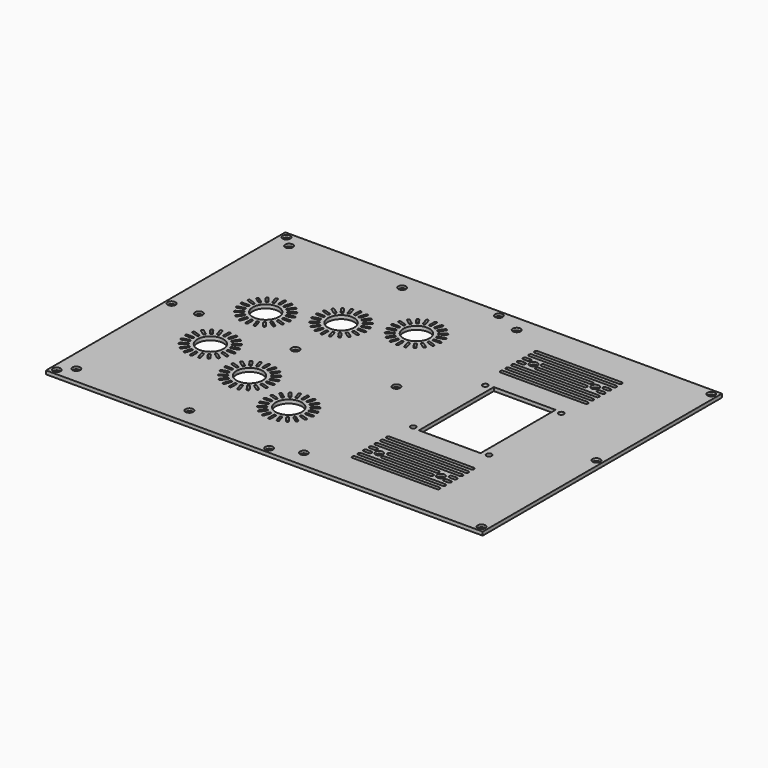
from build123d import *

# Parameters (mm, degrees)
F0_W           = 368
F0_H           = 252
F0_R           = 11
F0_R_2         = 2.25
F0_W_2         = 52
F0_H_2         = 79
F1_DEPTH       = 3
F2_D           = 3.5
F2_CBORE_D     = 6.5
F2_CBORE_DEPTH = 2
F4_D           = 3.5
F4_CBORE_D     = 6.5
F4_CBORE_DEPTH = 2
F6_DEPTH       = 3.001
F8_D           = 3.5
F8_CBORE_D     = 6.5
F8_CBORE_DEPTH = 2


# Not quite as in the source:
# - a feature names something its author has since deleted; it is built from what else it names


with BuildPart() as f1:
    # F0 (on Top) → F1 (new body)
    with BuildSketch(Plane.XY):
        Rectangle(F0_W, F0_H)
        with BuildLine():
            ThreePointArc((-79.0662379212, -61.5247912281), (-78.4842483914, -62.0218572447), (-78.4241983993, -62.7848647388))
            Line((-78.4241983993, -62.7848647388), (-79.9692833712, -67.5401473203))
            ThreePointArc((-79.9692833712, -67.5401473203), (-80.4663493878, -68.1221368501), (-81.2293568819, -68.1821868422))
            ThreePointArc((-81.2293568819, -68.1821868422), (-81.8113464117, -67.6851208256), (-81.8713964038, -66.9221133315))
            Line((-81.8713964038, -66.9221133315), (-80.3263114319, -62.1668307501))
            ThreePointArc((-80.3263114319, -62.1668307501), (-79.8292454154, -61.5848412202), (-79.0662379212, -61.5247912281))
        make_face(mode=Mode.SUBTRACT)
        with BuildLine():
            ThreePointArc((-74.74, -62.21), (-74.0328932188, -62.5028932188), (-73.74, -63.21))
            Line((-73.74, -63.21), (-73.74, -68.21))
            ThreePointArc((-73.74, -68.21), (-74.0328932188, -68.9171067812), (-74.74, -69.21))
            ThreePointArc((-74.74, -69.21), (-75.4471067812, -68.9171067812), (-75.74, -68.21))
            Line((-75.74, -68.21), (-75.74, -63.21))
            ThreePointArc((-75.74, -63.21), (-75.4471067812, -62.5028932188), (-74.74, -62.21))
        make_face(mode=Mode.SUBTRACT)
        with BuildLine():
            ThreePointArc((-70.4137620788, -61.5247912281), (-69.6507545846, -61.5848412202), (-69.1536885681, -62.1668307501))
            Line((-69.1536885681, -62.1668307501), (-67.6086035962, -66.9221133315))
            ThreePointArc((-67.6086035962, -66.9221133315), (-67.6686535883, -67.6851208256), (-68.2506431181, -68.1821868422))
            ThreePointArc((-68.2506431181, -68.1821868422), (-69.0136506122, -68.1221368501), (-69.5107166288, -67.5401473203))
            Line((-69.5107166288, -67.5401473203), (-71.0558016007, -62.7848647388))
            ThreePointArc((-71.0558016007, -62.7848647388), (-70.9957516086, -62.0218572447), (-70.4137620788, -61.5247912281))
        make_face(mode=Mode.SUBTRACT)
        with BuildLine():
            ThreePointArc((-38.8234902981, -84.2493568819), (-39.2233933864, -83.5967743525), (-39.0447220402, -82.8525546352))
            Line((-39.0447220402, -82.8525546352), (-36.1057957788, -78.8074696633))
            ThreePointArc((-36.1057957788, -78.8074696633), (-35.4532132494, -78.407566575), (-34.7089935321, -78.5862379212))
            ThreePointArc((-34.7089935321, -78.5862379212), (-34.3090904438, -79.2388204506), (-34.48776179, -79.9830401679))
            Line((-34.48776179, -79.9830401679), (-37.4266880515, -84.0281251398))
            ThreePointArc((-37.4266880515, -84.0281251398), (-38.0792705808, -84.4280282281), (-38.8234902981, -84.2493568819))
        make_face(mode=Mode.SUBTRACT)
        with BuildLine():
            ThreePointArc((-32.9693568819, -87.2321868422), (-33.5513464117, -86.7351208256), (-33.6113964038, -85.9721133315))
            Line((-33.6113964038, -85.9721133315), (-32.0663114319, -81.2168307501))
            ThreePointArc((-32.0663114319, -81.2168307501), (-31.5692454154, -80.6348412202), (-30.8062379212, -80.5747912281))
            ThreePointArc((-30.8062379212, -80.5747912281), (-30.2242483914, -81.0718572447), (-30.1641983993, -81.8348647388))
            Line((-30.1641983993, -81.8348647388), (-31.7092833712, -86.5901473203))
            ThreePointArc((-31.7092833712, -86.5901473203), (-32.2063493878, -87.1721368501), (-32.9693568819, -87.2321868422))
        make_face(mode=Mode.SUBTRACT)
        with BuildLine():
            ThreePointArc((-26.48, -88.26), (-27.1871067812, -87.9671067812), (-27.48, -87.26))
            Line((-27.48, -87.26), (-27.48, -82.26))
            ThreePointArc((-27.48, -82.26), (-27.1871067812, -81.5528932188), (-26.48, -81.26))
            ThreePointArc((-26.48, -81.26), (-25.7728932188, -81.5528932188), (-25.48, -82.26))
            Line((-25.48, -82.26), (-25.48, -87.26))
            ThreePointArc((-25.48, -87.26), (-25.7728932188, -87.9671067812), (-26.48, -88.26))
        make_face(mode=Mode.SUBTRACT)
        with BuildLine():
            ThreePointArc((-19.9906431181, -87.2321868422), (-20.7536506122, -87.1721368501), (-21.2507166288, -86.5901473203))
            Line((-21.2507166288, -86.5901473203), (-22.7958016007, -81.8348647388))
            ThreePointArc((-22.7958016007, -81.8348647388), (-22.7357516086, -81.0718572447), (-22.1537620788, -80.5747912281))
            ThreePointArc((-22.1537620788, -80.5747912281), (-21.3907545846, -80.6348412202), (-20.8936885681, -81.2168307501))
            Line((-20.8936885681, -81.2168307501), (-19.3486035962, -85.9721133315))
            ThreePointArc((-19.3486035962, -85.9721133315), (-19.4086535883, -86.7351208256), (-19.9906431181, -87.2321868422))
        make_face(mode=Mode.SUBTRACT)
        with BuildLine():
            ThreePointArc((-14.1365097019, -84.2493568819), (-14.8807294192, -84.4280282281), (-15.5333119485, -84.0281251398))
            Line((-15.5333119485, -84.0281251398), (-18.47223821, -79.9830401679))
            ThreePointArc((-18.47223821, -79.9830401679), (-18.6509095562, -79.2388204506), (-18.2510064679, -78.5862379212))
            ThreePointArc((-18.2510064679, -78.5862379212), (-17.5067867506, -78.407566575), (-16.8542042212, -78.8074696633))
            Line((-16.8542042212, -78.8074696633), (-13.9152779598, -82.8525546352))
            ThreePointArc((-13.9152779598, -82.8525546352), (-13.7366066136, -83.5967743525), (-14.1365097019, -84.2493568819))
        make_face(mode=Mode.SUBTRACT)
        with BuildLine():
            ThreePointArc((-43.4693568819, -79.6034902981), (-43.6480282281, -78.8592705808), (-43.2481251398, -78.2066880515))
            Line((-43.2481251398, -78.2066880515), (-39.2030401679, -75.26776179))
            ThreePointArc((-39.2030401679, -75.26776179), (-38.4588204506, -75.0890904438), (-37.8062379212, -75.4889935321))
            ThreePointArc((-37.8062379212, -75.4889935321), (-37.627566575, -76.2332132494), (-38.0274696633, -76.8857957788))
            Line((-38.0274696633, -76.8857957788), (-42.0725546352, -79.8247220402))
            ThreePointArc((-42.0725546352, -79.8247220402), (-42.8167743525, -80.0033933864), (-43.4693568819, -79.6034902981))
        make_face(mode=Mode.SUBTRACT)
        with BuildLine():
            ThreePointArc((-46.4521868422, -73.7493568819), (-46.3921368501, -72.9863493878), (-45.8101473203, -72.4892833712))
            Line((-45.8101473203, -72.4892833712), (-41.0548647388, -70.9441983993))
            ThreePointArc((-41.0548647388, -70.9441983993), (-40.2918572447, -71.0042483914), (-39.7947912281, -71.5862379212))
            ThreePointArc((-39.7947912281, -71.5862379212), (-39.8548412202, -72.3492454154), (-40.4368307501, -72.8463114319))
            Line((-40.4368307501, -72.8463114319), (-45.1921133315, -74.3913964038))
            ThreePointArc((-45.1921133315, -74.3913964038), (-45.9551208256, -74.3313464117), (-46.4521868422, -73.7493568819))
        make_face(mode=Mode.SUBTRACT)
        with BuildLine():
            ThreePointArc((-47.48, -67.26), (-47.1871067812, -66.5528932188), (-46.48, -66.26))
            Line((-46.48, -66.26), (-41.48, -66.26))
            ThreePointArc((-41.48, -66.26), (-40.7728932188, -66.5528932188), (-40.48, -67.26))
            ThreePointArc((-40.48, -67.26), (-40.7728932188, -67.9671067812), (-41.48, -68.26))
            Line((-41.48, -68.26), (-46.48, -68.26))
            ThreePointArc((-46.48, -68.26), (-47.1871067812, -67.9671067812), (-47.48, -67.26))
        make_face(mode=Mode.SUBTRACT)
        with Locations((-26.48, -67.26)):
            Circle(F0_R, mode=Mode.SUBTRACT)
        with BuildLine():
            ThreePointArc((-9.4906431181, -79.6034902981), (-10.1432256475, -80.0033933864), (-10.8874453648, -79.8247220402))
            Line((-10.8874453648, -79.8247220402), (-14.9325303367, -76.8857957788))
            ThreePointArc((-14.9325303367, -76.8857957788), (-15.332433425, -76.2332132494), (-15.1537620788, -75.4889935321))
            ThreePointArc((-15.1537620788, -75.4889935321), (-14.5011795494, -75.0890904438), (-13.7569598321, -75.26776179))
            Line((-13.7569598321, -75.26776179), (-9.7118748602, -78.2066880515))
            ThreePointArc((-9.7118748602, -78.2066880515), (-9.3119717719, -78.8592705808), (-9.4906431181, -79.6034902981))
        make_face(mode=Mode.SUBTRACT)
        with BuildLine():
            ThreePointArc((-6.5078131578, -73.7493568819), (-7.0048791744, -74.3313464117), (-7.7678866685, -74.3913964038))
            Line((-7.7678866685, -74.3913964038), (-12.5231692499, -72.8463114319))
            ThreePointArc((-12.5231692499, -72.8463114319), (-13.1051587798, -72.3492454154), (-13.1652087719, -71.5862379212))
            ThreePointArc((-13.1652087719, -71.5862379212), (-12.6681427553, -71.0042483914), (-11.9051352612, -70.9441983993))
            Line((-11.9051352612, -70.9441983993), (-7.1498526797, -72.4892833712))
            ThreePointArc((-7.1498526797, -72.4892833712), (-6.5678631499, -72.9863493878), (-6.5078131578, -73.7493568819))
        make_face(mode=Mode.SUBTRACT)
        with BuildLine():
            ThreePointArc((-5.48, -67.26), (-5.7728932188, -67.9671067812), (-6.48, -68.26))
            Line((-6.48, -68.26), (-11.48, -68.26))
            ThreePointArc((-11.48, -68.26), (-12.1871067812, -67.9671067812), (-12.48, -67.26))
            ThreePointArc((-12.48, -67.26), (-12.1871067812, -66.5528932188), (-11.48, -66.26))
            Line((-11.48, -66.26), (-6.48, -66.26))
            ThreePointArc((-6.48, -66.26), (-5.7728932188, -66.5528932188), (-5.48, -67.26))
        make_face(mode=Mode.SUBTRACT)
        with BuildLine():
            Line((-136.9568307501, -34.7463114319), (-141.7121133315, -36.2913964038))
            ThreePointArc((-141.7121133315, -36.2913964038), (-142.4751208256, -36.2313464117), (-142.9721868422, -35.6493568819))
            ThreePointArc((-142.9721868422, -35.6493568819), (-142.9121368501, -34.8863493878), (-142.3301473203, -34.3892833712))
            Line((-142.3301473203, -34.3892833712), (-137.5748647388, -32.8441983993))
            ThreePointArc((-137.5748647388, -32.8441983993), (-136.8118572447, -32.9042483914), (-136.3147912281, -33.4862379212))
            ThreePointArc((-136.3147912281, -33.4862379212), (-136.3748412202, -34.2492454154), (-136.9568307501, -34.7463114319))
        make_face(mode=Mode.SUBTRACT)
        with BuildLine():
            ThreePointArc((-88.74, -48.21), (-89.0328932188, -48.9171067812), (-89.74, -49.21))
            Line((-89.74, -49.21), (-94.74, -49.21))
            ThreePointArc((-94.74, -49.21), (-95.4471067812, -48.9171067812), (-95.74, -48.21))
            ThreePointArc((-95.74, -48.21), (-95.4471067812, -47.5028932188), (-94.74, -47.21))
            Line((-94.74, -47.21), (-89.74, -47.21))
            ThreePointArc((-89.74, -47.21), (-89.0328932188, -47.5028932188), (-88.74, -48.21))
        make_face(mode=Mode.SUBTRACT)
        with BuildLine():
            Line((-131.00776179, -41.8830401679), (-133.9466880515, -45.9281251398))
            ThreePointArc((-133.9466880515, -45.9281251398), (-134.5992705808, -46.3280282281), (-135.3434902981, -46.1493568819))
            ThreePointArc((-135.3434902981, -46.1493568819), (-135.7433933864, -45.4967743525), (-135.5647220402, -44.7525546352))
            Line((-135.5647220402, -44.7525546352), (-132.6257957788, -40.7074696633))
            ThreePointArc((-132.6257957788, -40.7074696633), (-131.9732132494, -40.307566575), (-131.2289935321, -40.4862379212))
            ThreePointArc((-131.2289935321, -40.4862379212), (-130.8290904438, -41.1388204506), (-131.00776179, -41.8830401679))
        make_face(mode=Mode.SUBTRACT)
        with BuildLine():
            Line((-126.6841983993, -43.7348647388), (-128.2292833712, -48.4901473203))
            ThreePointArc((-128.2292833712, -48.4901473203), (-128.7263493878, -49.0721368501), (-129.4893568819, -49.1321868422))
            ThreePointArc((-129.4893568819, -49.1321868422), (-130.0713464117, -48.6351208256), (-130.1313964038, -47.8721133315))
            Line((-130.1313964038, -47.8721133315), (-128.5863114319, -43.1168307501))
            ThreePointArc((-128.5863114319, -43.1168307501), (-128.0892454154, -42.5348412202), (-127.3262379212, -42.4747912281))
            ThreePointArc((-127.3262379212, -42.4747912281), (-126.7442483914, -42.9718572447), (-126.6841983993, -43.7348647388))
        make_face(mode=Mode.SUBTRACT)
        with BuildLine():
            Line((-134.5474696633, -38.7857957788), (-138.5925546352, -41.7247220402))
            ThreePointArc((-138.5925546352, -41.7247220402), (-139.3367743525, -41.9033933864), (-139.9893568819, -41.5034902981))
            ThreePointArc((-139.9893568819, -41.5034902981), (-140.1680282281, -40.7592705808), (-139.7681251398, -40.1066880515))
            Line((-139.7681251398, -40.1066880515), (-135.7230401679, -37.16776179))
            ThreePointArc((-135.7230401679, -37.16776179), (-134.9788204506, -36.9890904438), (-134.3262379212, -37.3889935321))
            ThreePointArc((-134.3262379212, -37.3889935321), (-134.147566575, -38.1332132494), (-134.5474696633, -38.7857957788))
        make_face(mode=Mode.SUBTRACT)
        with BuildLine():
            Line((-122, -44.16), (-122, -49.16))
            ThreePointArc((-122, -49.16), (-122.2928932188, -49.8671067812), (-123, -50.16))
            ThreePointArc((-123, -50.16), (-123.7071067812, -49.8671067812), (-124, -49.16))
            Line((-124, -49.16), (-124, -44.16))
            ThreePointArc((-124, -44.16), (-123.7071067812, -43.4528932188), (-123, -43.16))
            ThreePointArc((-123, -43.16), (-122.2928932188, -43.4528932188), (-122, -44.16))
        make_face(mode=Mode.SUBTRACT)
        with BuildLine():
            Line((-117.4136885681, -43.1168307501), (-115.8686035962, -47.8721133315))
            ThreePointArc((-115.8686035962, -47.8721133315), (-115.9286535883, -48.6351208256), (-116.5106431181, -49.1321868422))
            ThreePointArc((-116.5106431181, -49.1321868422), (-117.2736506122, -49.0721368501), (-117.7707166288, -48.4901473203))
            Line((-117.7707166288, -48.4901473203), (-119.3158016007, -43.7348647388))
            ThreePointArc((-119.3158016007, -43.7348647388), (-119.2557516086, -42.9718572447), (-118.6737620788, -42.4747912281))
            ThreePointArc((-118.6737620788, -42.4747912281), (-117.9107545846, -42.5348412202), (-117.4136885681, -43.1168307501))
        make_face(mode=Mode.SUBTRACT)
        with BuildLine():
            Line((-113.3742042212, -40.7074696633), (-110.4352779598, -44.7525546352))
            ThreePointArc((-110.4352779598, -44.7525546352), (-110.2566066136, -45.4967743525), (-110.6565097019, -46.1493568819))
            ThreePointArc((-110.6565097019, -46.1493568819), (-111.4007294192, -46.3280282281), (-112.0533119485, -45.9281251398))
            Line((-112.0533119485, -45.9281251398), (-114.99223821, -41.8830401679))
            ThreePointArc((-114.99223821, -41.8830401679), (-115.1709095562, -41.1388204506), (-114.7710064679, -40.4862379212))
            ThreePointArc((-114.7710064679, -40.4862379212), (-114.0267867506, -40.307566575), (-113.3742042212, -40.7074696633))
        make_face(mode=Mode.SUBTRACT)
        with BuildLine():
            Line((-110.2769598321, -37.16776179), (-106.2318748602, -40.1066880515))
            ThreePointArc((-106.2318748602, -40.1066880515), (-105.8319717719, -40.7592705808), (-106.0106431181, -41.5034902981))
            ThreePointArc((-106.0106431181, -41.5034902981), (-106.6632256475, -41.9033933864), (-107.4074453648, -41.7247220402))
            Line((-107.4074453648, -41.7247220402), (-111.4525303367, -38.7857957788))
            ThreePointArc((-111.4525303367, -38.7857957788), (-111.852433425, -38.1332132494), (-111.6737620788, -37.3889935321))
            ThreePointArc((-111.6737620788, -37.3889935321), (-111.0211795494, -36.9890904438), (-110.2769598321, -37.16776179))
        make_face(mode=Mode.SUBTRACT)
        with BuildLine():
            Line((-108.4251352612, -32.8441983993), (-103.6698526797, -34.3892833712))
            ThreePointArc((-103.6698526797, -34.3892833712), (-103.0878631499, -34.8863493878), (-103.0278131578, -35.6493568819))
            ThreePointArc((-103.0278131578, -35.6493568819), (-103.5248791744, -36.2313464117), (-104.2878866685, -36.2913964038))
            Line((-104.2878866685, -36.2913964038), (-109.0431692499, -34.7463114319))
            ThreePointArc((-109.0431692499, -34.7463114319), (-109.6251587798, -34.2492454154), (-109.6852087719, -33.4862379212))
            ThreePointArc((-109.6852087719, -33.4862379212), (-109.1881427553, -32.9042483914), (-108.4251352612, -32.8441983993))
        make_face(mode=Mode.SUBTRACT)
        with BuildLine():
            Line((-138, -30.16), (-143, -30.16))
            ThreePointArc((-143, -30.16), (-143.7071067812, -29.8671067812), (-144, -29.16))
            ThreePointArc((-144, -29.16), (-143.7071067812, -28.4528932188), (-143, -28.16))
            Line((-143, -28.16), (-138, -28.16))
            ThreePointArc((-138, -28.16), (-137.2928932188, -28.4528932188), (-137, -29.16))
            ThreePointArc((-137, -29.16), (-137.2928932188, -29.8671067812), (-138, -30.16))
        make_face(mode=Mode.SUBTRACT)
        with BuildLine():
            Line((-137.5748647388, -25.4758016007), (-142.3301473203, -23.9307166288))
            ThreePointArc((-142.3301473203, -23.9307166288), (-142.9121368501, -23.4336506122), (-142.9721868422, -22.6706431181))
            ThreePointArc((-142.9721868422, -22.6706431181), (-142.4751208256, -22.0886535883), (-141.7121133315, -22.0286035962))
            Line((-141.7121133315, -22.0286035962), (-136.9568307501, -23.5736885681))
            ThreePointArc((-136.9568307501, -23.5736885681), (-136.3748412202, -24.0707545846), (-136.3147912281, -24.8337620788))
            ThreePointArc((-136.3147912281, -24.8337620788), (-136.8118572447, -25.4157516086), (-137.5748647388, -25.4758016007))
        make_face(mode=Mode.SUBTRACT)
        with Locations((-123, -29.16)):
            Circle(F0_R, mode=Mode.SUBTRACT)
        with BuildLine():
            Line((-135.7230401679, -21.15223821), (-139.7681251398, -18.2133119485))
            ThreePointArc((-139.7681251398, -18.2133119485), (-140.1680282281, -17.5607294192), (-139.9893568819, -16.8165097019))
            ThreePointArc((-139.9893568819, -16.8165097019), (-139.3367743525, -16.4166066136), (-138.5925546352, -16.5952779598))
            Line((-138.5925546352, -16.5952779598), (-134.5474696633, -19.5342042212))
            ThreePointArc((-134.5474696633, -19.5342042212), (-134.147566575, -20.1867867506), (-134.3262379212, -20.9310064679))
            ThreePointArc((-134.3262379212, -20.9310064679), (-134.9788204506, -21.3309095562), (-135.7230401679, -21.15223821))
        make_face(mode=Mode.SUBTRACT)
        with BuildLine():
            Line((-108, -28.16), (-103, -28.16))
            ThreePointArc((-103, -28.16), (-102.2928932188, -28.4528932188), (-102, -29.16))
            ThreePointArc((-102, -29.16), (-102.2928932188, -29.8671067812), (-103, -30.16))
            Line((-103, -30.16), (-108, -30.16))
            ThreePointArc((-108, -30.16), (-108.7071067812, -29.8671067812), (-109, -29.16))
            ThreePointArc((-109, -29.16), (-108.7071067812, -28.4528932188), (-108, -28.16))
        make_face(mode=Mode.SUBTRACT)
        with BuildLine():
            Line((-109.0431692499, -23.5736885681), (-104.2878866685, -22.0286035962))
            ThreePointArc((-104.2878866685, -22.0286035962), (-103.5248791744, -22.0886535883), (-103.0278131578, -22.6706431181))
            ThreePointArc((-103.0278131578, -22.6706431181), (-103.0878631499, -23.4336506122), (-103.6698526797, -23.9307166288))
            Line((-103.6698526797, -23.9307166288), (-108.4251352612, -25.4758016007))
            ThreePointArc((-108.4251352612, -25.4758016007), (-109.1881427553, -25.4157516086), (-109.6852087719, -24.8337620788))
            ThreePointArc((-109.6852087719, -24.8337620788), (-109.6251587798, -24.0707545846), (-109.0431692499, -23.5736885681))
        make_face(mode=Mode.SUBTRACT)
        with BuildLine():
            Line((-111.4525303367, -19.5342042212), (-107.4074453648, -16.5952779598))
            ThreePointArc((-107.4074453648, -16.5952779598), (-106.6632256475, -16.4166066136), (-106.0106431181, -16.8165097019))
            ThreePointArc((-106.0106431181, -16.8165097019), (-105.8319717719, -17.5607294192), (-106.2318748602, -18.2133119485))
            Line((-106.2318748602, -18.2133119485), (-110.2769598321, -21.15223821))
            ThreePointArc((-110.2769598321, -21.15223821), (-111.0211795494, -21.3309095562), (-111.6737620788, -20.9310064679))
            ThreePointArc((-111.6737620788, -20.9310064679), (-111.852433425, -20.1867867506), (-111.4525303367, -19.5342042212))
        make_face(mode=Mode.SUBTRACT)
        with BuildLine():
            Line((-132.6257957788, -17.6125303367), (-135.5647220402, -13.5674453648))
            ThreePointArc((-135.5647220402, -13.5674453648), (-135.7433933864, -12.8232256475), (-135.3434902981, -12.1706431181))
            ThreePointArc((-135.3434902981, -12.1706431181), (-134.5992705808, -11.9919717719), (-133.9466880515, -12.3918748602))
            Line((-133.9466880515, -12.3918748602), (-131.00776179, -16.4369598321))
            ThreePointArc((-131.00776179, -16.4369598321), (-130.8290904438, -17.1811795494), (-131.2289935321, -17.8337620788))
            ThreePointArc((-131.2289935321, -17.8337620788), (-131.9732132494, -18.012433425), (-132.6257957788, -17.6125303367))
        make_face(mode=Mode.SUBTRACT)
        with BuildLine():
            Line((-128.5863114319, -15.2031692499), (-130.1313964038, -10.4478866685))
            ThreePointArc((-130.1313964038, -10.4478866685), (-130.0713464117, -9.6848791744), (-129.4893568819, -9.1878131578))
            ThreePointArc((-129.4893568819, -9.1878131578), (-128.7263493878, -9.2478631499), (-128.2292833712, -9.8298526797))
            Line((-128.2292833712, -9.8298526797), (-126.6841983993, -14.5851352612))
            ThreePointArc((-126.6841983993, -14.5851352612), (-126.7442483914, -15.3481427553), (-127.3262379212, -15.8452087719))
            ThreePointArc((-127.3262379212, -15.8452087719), (-128.0892454154, -15.7851587798), (-128.5863114319, -15.2031692499))
        make_face(mode=Mode.SUBTRACT)
        with BuildLine():
            Line((-119.3158016007, -14.5851352612), (-117.7707166288, -9.8298526797))
            ThreePointArc((-117.7707166288, -9.8298526797), (-117.2736506122, -9.2478631499), (-116.5106431181, -9.1878131578))
            ThreePointArc((-116.5106431181, -9.1878131578), (-115.9286535883, -9.6848791744), (-115.8686035962, -10.4478866685))
            Line((-115.8686035962, -10.4478866685), (-117.4136885681, -15.2031692499))
            ThreePointArc((-117.4136885681, -15.2031692499), (-117.9107545846, -15.7851587798), (-118.6737620788, -15.8452087719))
            ThreePointArc((-118.6737620788, -15.8452087719), (-119.2557516086, -15.3481427553), (-119.3158016007, -14.5851352612))
        make_face(mode=Mode.SUBTRACT)
        with BuildLine():
            Line((-124, -14.16), (-124, -9.16))
            ThreePointArc((-124, -9.16), (-123.7071067812, -8.4528932188), (-123, -8.16))
            ThreePointArc((-123, -8.16), (-122.2928932188, -8.4528932188), (-122, -9.16))
            Line((-122, -9.16), (-122, -14.16))
            ThreePointArc((-122, -14.16), (-122.2928932188, -14.8671067812), (-123, -15.16))
            ThreePointArc((-123, -15.16), (-123.7071067812, -14.8671067812), (-124, -14.16))
        make_face(mode=Mode.SUBTRACT)
        with BuildLine():
            Line((-114.99223821, -16.4369598321), (-112.0533119485, -12.3918748602))
            ThreePointArc((-112.0533119485, -12.3918748602), (-111.4007294192, -11.9919717719), (-110.6565097019, -12.1706431181))
            ThreePointArc((-110.6565097019, -12.1706431181), (-110.2566066136, -12.8232256475), (-110.4352779598, -13.5674453648))
            Line((-110.4352779598, -13.5674453648), (-113.3742042212, -17.6125303367))
            ThreePointArc((-113.3742042212, -17.6125303367), (-114.0267867506, -18.012433425), (-114.7710064679, -17.8337620788))
            ThreePointArc((-114.7710064679, -17.8337620788), (-115.1709095562, -17.1811795494), (-114.99223821, -16.4369598321))
        make_face(mode=Mode.SUBTRACT)
        with BuildLine():
            ThreePointArc((-82.9689935321, -59.5362379212), (-82.5690904438, -60.1888204506), (-82.74776179, -60.9330401679))
            Line((-82.74776179, -60.9330401679), (-85.6866880515, -64.9781251398))
            ThreePointArc((-85.6866880515, -64.9781251398), (-86.3392705808, -65.3780282281), (-87.0834902981, -65.1993568819))
            ThreePointArc((-87.0834902981, -65.1993568819), (-87.4833933864, -64.5467743525), (-87.3047220402, -63.8025546352))
            Line((-87.3047220402, -63.8025546352), (-84.3657957788, -59.7574696633))
            ThreePointArc((-84.3657957788, -59.7574696633), (-83.7132132494, -59.357566575), (-82.9689935321, -59.5362379212))
        make_face(mode=Mode.SUBTRACT)
        with BuildLine():
            ThreePointArc((-86.0662379212, -56.4389935321), (-85.887566575, -57.1832132494), (-86.2874696633, -57.8357957788))
            Line((-86.2874696633, -57.8357957788), (-90.3325546352, -60.7747220402))
            ThreePointArc((-90.3325546352, -60.7747220402), (-91.0767743525, -60.9533933864), (-91.7293568819, -60.5534902981))
            ThreePointArc((-91.7293568819, -60.5534902981), (-91.9080282281, -59.8092705808), (-91.5081251398, -59.1566880515))
            Line((-91.5081251398, -59.1566880515), (-87.4630401679, -56.21776179))
            ThreePointArc((-87.4630401679, -56.21776179), (-86.7188204506, -56.0390904438), (-86.0662379212, -56.4389935321))
        make_face(mode=Mode.SUBTRACT)
        with BuildLine():
            ThreePointArc((-88.0547912281, -52.5362379212), (-88.1148412202, -53.2992454154), (-88.6968307501, -53.7963114319))
            Line((-88.6968307501, -53.7963114319), (-93.4521133315, -55.3413964038))
            ThreePointArc((-93.4521133315, -55.3413964038), (-94.2151208256, -55.2813464117), (-94.7121868422, -54.6993568819))
            ThreePointArc((-94.7121868422, -54.6993568819), (-94.6521368501, -53.9363493878), (-94.0701473203, -53.4392833712))
            Line((-94.0701473203, -53.4392833712), (-89.3148647388, -51.8941983993))
            ThreePointArc((-89.3148647388, -51.8941983993), (-88.5518572447, -51.9542483914), (-88.0547912281, -52.5362379212))
        make_face(mode=Mode.SUBTRACT)
        with Locations((-74.74, -48.21)):
            Circle(F0_R, mode=Mode.SUBTRACT)
        with BuildLine():
            ThreePointArc((-66.5110064679, -59.5362379212), (-65.7667867506, -59.357566575), (-65.1142042212, -59.7574696633))
            Line((-65.1142042212, -59.7574696633), (-62.1752779598, -63.8025546352))
            ThreePointArc((-62.1752779598, -63.8025546352), (-61.9966066136, -64.5467743525), (-62.3965097019, -65.1993568819))
            ThreePointArc((-62.3965097019, -65.1993568819), (-63.1407294192, -65.3780282281), (-63.7933119485, -64.9781251398))
            Line((-63.7933119485, -64.9781251398), (-66.73223821, -60.9330401679))
            ThreePointArc((-66.73223821, -60.9330401679), (-66.9109095562, -60.1888204506), (-66.5110064679, -59.5362379212))
        make_face(mode=Mode.SUBTRACT)
        with BuildLine():
            ThreePointArc((-63.4137620788, -56.4389935321), (-62.7611795494, -56.0390904438), (-62.0169598321, -56.21776179))
            Line((-62.0169598321, -56.21776179), (-57.9718748602, -59.1566880515))
            ThreePointArc((-57.9718748602, -59.1566880515), (-57.5719717719, -59.8092705808), (-57.7506431181, -60.5534902981))
            ThreePointArc((-57.7506431181, -60.5534902981), (-58.4032256475, -60.9533933864), (-59.1474453648, -60.7747220402))
            Line((-59.1474453648, -60.7747220402), (-63.1925303367, -57.8357957788))
            ThreePointArc((-63.1925303367, -57.8357957788), (-63.592433425, -57.1832132494), (-63.4137620788, -56.4389935321))
        make_face(mode=Mode.SUBTRACT)
        with BuildLine():
            ThreePointArc((-61.4252087719, -52.5362379212), (-60.9281427553, -51.9542483914), (-60.1651352612, -51.8941983993))
            Line((-60.1651352612, -51.8941983993), (-55.4098526797, -53.4392833712))
            ThreePointArc((-55.4098526797, -53.4392833712), (-54.8278631499, -53.9363493878), (-54.7678131578, -54.6993568819))
            ThreePointArc((-54.7678131578, -54.6993568819), (-55.2648791744, -55.2813464117), (-56.0278866685, -55.3413964038))
            Line((-56.0278866685, -55.3413964038), (-60.7831692499, -53.7963114319))
            ThreePointArc((-60.7831692499, -53.7963114319), (-61.3651587798, -53.2992454154), (-61.4252087719, -52.5362379212))
        make_face(mode=Mode.SUBTRACT)
        with BuildLine():
            ThreePointArc((-60.74, -48.21), (-60.4471067812, -47.5028932188), (-59.74, -47.21))
            Line((-59.74, -47.21), (-54.74, -47.21))
            ThreePointArc((-54.74, -47.21), (-54.0328932188, -47.5028932188), (-53.74, -48.21))
            ThreePointArc((-53.74, -48.21), (-54.0328932188, -48.9171067812), (-54.74, -49.21))
            Line((-54.74, -49.21), (-59.74, -49.21))
            ThreePointArc((-59.74, -49.21), (-60.4471067812, -48.9171067812), (-60.74, -48.21))
        make_face(mode=Mode.SUBTRACT)
        with BuildLine():
            ThreePointArc((-88.0547912281, -43.8837620788), (-88.5518572447, -44.4657516086), (-89.3148647388, -44.5258016007))
            Line((-89.3148647388, -44.5258016007), (-94.0701473203, -42.9807166288))
            ThreePointArc((-94.0701473203, -42.9807166288), (-94.6521368501, -42.4836506122), (-94.7121868422, -41.7206431181))
            ThreePointArc((-94.7121868422, -41.7206431181), (-94.2151208256, -41.1386535883), (-93.4521133315, -41.0786035962))
            Line((-93.4521133315, -41.0786035962), (-88.6968307501, -42.6236885681))
            ThreePointArc((-88.6968307501, -42.6236885681), (-88.1148412202, -43.1207545846), (-88.0547912281, -43.8837620788))
        make_face(mode=Mode.SUBTRACT)
        with BuildLine():
            ThreePointArc((-86.0662379212, -39.9810064679), (-86.7188204506, -40.3809095562), (-87.4630401679, -40.20223821))
            Line((-87.4630401679, -40.20223821), (-91.5081251398, -37.2633119485))
            ThreePointArc((-91.5081251398, -37.2633119485), (-91.9080282281, -36.6107294192), (-91.7293568819, -35.8665097019))
            ThreePointArc((-91.7293568819, -35.8665097019), (-91.0767743525, -35.4666066136), (-90.3325546352, -35.6452779598))
            Line((-90.3325546352, -35.6452779598), (-86.2874696633, -38.5842042212))
            ThreePointArc((-86.2874696633, -38.5842042212), (-85.887566575, -39.2367867506), (-86.0662379212, -39.9810064679))
        make_face(mode=Mode.SUBTRACT)
        with BuildLine():
            ThreePointArc((-82.9689935321, -36.8837620788), (-83.7132132494, -37.062433425), (-84.3657957788, -36.6625303367))
            Line((-84.3657957788, -36.6625303367), (-87.3047220402, -32.6174453648))
            ThreePointArc((-87.3047220402, -32.6174453648), (-87.4833933864, -31.8732256475), (-87.0834902981, -31.2206431181))
            ThreePointArc((-87.0834902981, -31.2206431181), (-86.3392705808, -31.0419717719), (-85.6866880515, -31.4418748602))
            Line((-85.6866880515, -31.4418748602), (-82.74776179, -35.4869598321))
            ThreePointArc((-82.74776179, -35.4869598321), (-82.5690904438, -36.2311795494), (-82.9689935321, -36.8837620788))
        make_face(mode=Mode.SUBTRACT)
        with BuildLine():
            ThreePointArc((-79.0662379212, -34.8952087719), (-79.8292454154, -34.8351587798), (-80.3263114319, -34.2531692499))
            Line((-80.3263114319, -34.2531692499), (-81.8713964038, -29.4978866685))
            ThreePointArc((-81.8713964038, -29.4978866685), (-81.8113464117, -28.7348791744), (-81.2293568819, -28.2378131578))
            ThreePointArc((-81.2293568819, -28.2378131578), (-80.4663493878, -28.2978631499), (-79.9692833712, -28.8798526797))
            Line((-79.9692833712, -28.8798526797), (-78.4241983993, -33.6351352612))
            ThreePointArc((-78.4241983993, -33.6351352612), (-78.4842483914, -34.3981427553), (-79.0662379212, -34.8952087719))
        make_face(mode=Mode.SUBTRACT)
        with BuildLine():
            ThreePointArc((-70.4137620788, -34.8952087719), (-70.9957516086, -34.3981427553), (-71.0558016007, -33.6351352612))
            Line((-71.0558016007, -33.6351352612), (-69.5107166288, -28.8798526797))
            ThreePointArc((-69.5107166288, -28.8798526797), (-69.0136506122, -28.2978631499), (-68.2506431181, -28.2378131578))
            ThreePointArc((-68.2506431181, -28.2378131578), (-67.6686535883, -28.7348791744), (-67.6086035962, -29.4978866685))
            Line((-67.6086035962, -29.4978866685), (-69.1536885681, -34.2531692499))
            ThreePointArc((-69.1536885681, -34.2531692499), (-69.6507545846, -34.8351587798), (-70.4137620788, -34.8952087719))
        make_face(mode=Mode.SUBTRACT)
        with BuildLine():
            ThreePointArc((-61.4252087719, -43.8837620788), (-61.3651587798, -43.1207545846), (-60.7831692499, -42.6236885681))
            Line((-60.7831692499, -42.6236885681), (-56.0278866685, -41.0786035962))
            ThreePointArc((-56.0278866685, -41.0786035962), (-55.2648791744, -41.1386535883), (-54.7678131578, -41.7206431181))
            ThreePointArc((-54.7678131578, -41.7206431181), (-54.8278631499, -42.4836506122), (-55.4098526797, -42.9807166288))
            Line((-55.4098526797, -42.9807166288), (-60.1651352612, -44.5258016007))
            ThreePointArc((-60.1651352612, -44.5258016007), (-60.9281427553, -44.4657516086), (-61.4252087719, -43.8837620788))
        make_face(mode=Mode.SUBTRACT)
        with BuildLine():
            ThreePointArc((-63.4137620788, -39.9810064679), (-63.592433425, -39.2367867506), (-63.1925303367, -38.5842042212))
            Line((-63.1925303367, -38.5842042212), (-59.1474453648, -35.6452779598))
            ThreePointArc((-59.1474453648, -35.6452779598), (-58.4032256475, -35.4666066136), (-57.7506431181, -35.8665097019))
            ThreePointArc((-57.7506431181, -35.8665097019), (-57.5719717719, -36.6107294192), (-57.9718748602, -37.2633119485))
            Line((-57.9718748602, -37.2633119485), (-62.0169598321, -40.20223821))
            ThreePointArc((-62.0169598321, -40.20223821), (-62.7611795494, -40.3809095562), (-63.4137620788, -39.9810064679))
        make_face(mode=Mode.SUBTRACT)
        with BuildLine():
            ThreePointArc((-66.5110064679, -36.8837620788), (-66.9109095562, -36.2311795494), (-66.73223821, -35.4869598321))
            Line((-66.73223821, -35.4869598321), (-63.7933119485, -31.4418748602))
            ThreePointArc((-63.7933119485, -31.4418748602), (-63.1407294192, -31.0419717719), (-62.3965097019, -31.2206431181))
            ThreePointArc((-62.3965097019, -31.2206431181), (-61.9966066136, -31.8732256475), (-62.1752779598, -32.6174453648))
            Line((-62.1752779598, -32.6174453648), (-65.1142042212, -36.6625303367))
            ThreePointArc((-65.1142042212, -36.6625303367), (-65.7667867506, -37.062433425), (-66.5110064679, -36.8837620788))
        make_face(mode=Mode.SUBTRACT)
        with BuildLine():
            ThreePointArc((-46.4521868422, -60.7706431181), (-45.9551208256, -60.1886535883), (-45.1921133315, -60.1286035962))
            Line((-45.1921133315, -60.1286035962), (-40.4368307501, -61.6736885681))
            ThreePointArc((-40.4368307501, -61.6736885681), (-39.8548412202, -62.1707545846), (-39.7947912281, -62.9337620788))
            ThreePointArc((-39.7947912281, -62.9337620788), (-40.2918572447, -63.5157516086), (-41.0548647388, -63.5758016007))
            Line((-41.0548647388, -63.5758016007), (-45.8101473203, -62.0307166288))
            ThreePointArc((-45.8101473203, -62.0307166288), (-46.3921368501, -61.5336506122), (-46.4521868422, -60.7706431181))
        make_face(mode=Mode.SUBTRACT)
        with BuildLine():
            ThreePointArc((-43.4693568819, -54.9165097019), (-42.8167743525, -54.5166066136), (-42.0725546352, -54.6952779598))
            Line((-42.0725546352, -54.6952779598), (-38.0274696633, -57.6342042212))
            ThreePointArc((-38.0274696633, -57.6342042212), (-37.627566575, -58.2867867506), (-37.8062379212, -59.0310064679))
            ThreePointArc((-37.8062379212, -59.0310064679), (-38.4588204506, -59.4309095562), (-39.2030401679, -59.25223821))
            Line((-39.2030401679, -59.25223821), (-43.2481251398, -56.3133119485))
            ThreePointArc((-43.2481251398, -56.3133119485), (-43.6480282281, -55.6607294192), (-43.4693568819, -54.9165097019))
        make_face(mode=Mode.SUBTRACT)
        with BuildLine():
            ThreePointArc((-38.8234902981, -50.2706431181), (-38.0792705808, -50.0919717719), (-37.4266880515, -50.4918748602))
            Line((-37.4266880515, -50.4918748602), (-34.48776179, -54.5369598321))
            ThreePointArc((-34.48776179, -54.5369598321), (-34.3090904438, -55.2811795494), (-34.7089935321, -55.9337620788))
            ThreePointArc((-34.7089935321, -55.9337620788), (-35.4532132494, -56.112433425), (-36.1057957788, -55.7125303367))
            Line((-36.1057957788, -55.7125303367), (-39.0447220402, -51.6674453648))
            ThreePointArc((-39.0447220402, -51.6674453648), (-39.2233933864, -50.9232256475), (-38.8234902981, -50.2706431181))
        make_face(mode=Mode.SUBTRACT)
        with BuildLine():
            ThreePointArc((-32.9693568819, -47.2878131578), (-32.2063493878, -47.3478631499), (-31.7092833712, -47.9298526797))
            Line((-31.7092833712, -47.9298526797), (-30.1641983993, -52.6851352612))
            ThreePointArc((-30.1641983993, -52.6851352612), (-30.2242483914, -53.4481427553), (-30.8062379212, -53.9452087719))
            ThreePointArc((-30.8062379212, -53.9452087719), (-31.5692454154, -53.8851587798), (-32.0663114319, -53.3031692499))
            Line((-32.0663114319, -53.3031692499), (-33.6113964038, -48.5478866685))
            ThreePointArc((-33.6113964038, -48.5478866685), (-33.5513464117, -47.7848791744), (-32.9693568819, -47.2878131578))
        make_face(mode=Mode.SUBTRACT)
        with BuildLine():
            Line((-27.48, -52.26), (-27.48, -47.26))
            ThreePointArc((-27.48, -47.26), (-27.1871067812, -46.5528932188), (-26.48, -46.26))
            ThreePointArc((-26.48, -46.26), (-25.7728932188, -46.5528932188), (-25.48, -47.26))
            Line((-25.48, -47.26), (-25.48, -52.26))
            ThreePointArc((-25.48, -52.26), (-25.7728932188, -52.9671067812), (-26.48, -53.26))
            ThreePointArc((-26.48, -53.26), (-27.1871067812, -52.9671067812), (-27.48, -52.26))
        make_face(mode=Mode.SUBTRACT)
        with BuildLine():
            ThreePointArc((-9.4906431181, -54.9165097019), (-9.3119717719, -55.6607294192), (-9.7118748602, -56.3133119485))
            Line((-9.7118748602, -56.3133119485), (-13.7569598321, -59.25223821))
            ThreePointArc((-13.7569598321, -59.25223821), (-14.5011795494, -59.4309095562), (-15.1537620788, -59.0310064679))
            ThreePointArc((-15.1537620788, -59.0310064679), (-15.332433425, -58.2867867506), (-14.9325303367, -57.6342042212))
            Line((-14.9325303367, -57.6342042212), (-10.8874453648, -54.6952779598))
            ThreePointArc((-10.8874453648, -54.6952779598), (-10.1432256475, -54.5166066136), (-9.4906431181, -54.9165097019))
        make_face(mode=Mode.SUBTRACT)
        with BuildLine():
            ThreePointArc((-6.5078131578, -60.7706431181), (-6.5678631499, -61.5336506122), (-7.1498526797, -62.0307166288))
            Line((-7.1498526797, -62.0307166288), (-11.9051352612, -63.5758016007))
            ThreePointArc((-11.9051352612, -63.5758016007), (-12.6681427553, -63.5157516086), (-13.1652087719, -62.9337620788))
            ThreePointArc((-13.1652087719, -62.9337620788), (-13.1051587798, -62.1707545846), (-12.5231692499, -61.6736885681))
            Line((-12.5231692499, -61.6736885681), (-7.7678866685, -60.1286035962))
            ThreePointArc((-7.7678866685, -60.1286035962), (-7.0048791744, -60.1886535883), (-6.5078131578, -60.7706431181))
        make_face(mode=Mode.SUBTRACT)
        with BuildLine():
            ThreePointArc((-14.1365097019, -50.2706431181), (-13.7366066136, -50.9232256475), (-13.9152779598, -51.6674453648))
            Line((-13.9152779598, -51.6674453648), (-16.8542042212, -55.7125303367))
            ThreePointArc((-16.8542042212, -55.7125303367), (-17.5067867506, -56.112433425), (-18.2510064679, -55.9337620788))
            ThreePointArc((-18.2510064679, -55.9337620788), (-18.6509095562, -55.2811795494), (-18.47223821, -54.5369598321))
            Line((-18.47223821, -54.5369598321), (-15.5333119485, -50.4918748602))
            ThreePointArc((-15.5333119485, -50.4918748602), (-14.8807294192, -50.0919717719), (-14.1365097019, -50.2706431181))
        make_face(mode=Mode.SUBTRACT)
        with BuildLine():
            ThreePointArc((-19.9906431181, -47.2878131578), (-19.4086535883, -47.7848791744), (-19.3486035962, -48.5478866685))
            Line((-19.3486035962, -48.5478866685), (-20.8936885681, -53.3031692499))
            ThreePointArc((-20.8936885681, -53.3031692499), (-21.3907545846, -53.8851587798), (-22.1537620788, -53.9452087719))
            ThreePointArc((-22.1537620788, -53.9452087719), (-22.7357516086, -53.4481427553), (-22.7958016007, -52.6851352612))
            Line((-22.7958016007, -52.6851352612), (-21.2507166288, -47.9298526797))
            ThreePointArc((-21.2507166288, -47.9298526797), (-20.7536506122, -47.3478631499), (-19.9906431181, -47.2878131578))
        make_face(mode=Mode.SUBTRACT)
        with BuildLine():
            Line((-75.74, -33.21), (-75.74, -28.21))
            ThreePointArc((-75.74, -28.21), (-75.4471067812, -27.5028932188), (-74.74, -27.21))
            ThreePointArc((-74.74, -27.21), (-74.0328932188, -27.5028932188), (-73.74, -28.21))
            Line((-73.74, -28.21), (-73.74, -33.21))
            ThreePointArc((-73.74, -33.21), (-74.0328932188, -33.9171067812), (-74.74, -34.21))
            ThreePointArc((-74.74, -34.21), (-75.4471067812, -33.9171067812), (-75.74, -33.21))
        make_face(mode=Mode.SUBTRACT)
        with Locations((55, -38)):
            Circle(F0_R_2, mode=Mode.SUBTRACT)
        with Locations((119, -38)):
            Circle(F0_R_2, mode=Mode.SUBTRACT)
        with BuildLine():
            ThreePointArc((-142.9721868422, 22.6706431181), (-142.9121368501, 23.4336506122), (-142.3301473203, 23.9307166288))
            Line((-142.3301473203, 23.9307166288), (-137.5748647388, 25.4758016007))
            ThreePointArc((-137.5748647388, 25.4758016007), (-136.8118572447, 25.4157516086), (-136.3147912281, 24.8337620788))
            ThreePointArc((-136.3147912281, 24.8337620788), (-136.3748412202, 24.0707545846), (-136.9568307501, 23.5736885681))
            Line((-136.9568307501, 23.5736885681), (-141.7121133315, 22.0286035962))
            ThreePointArc((-141.7121133315, 22.0286035962), (-142.4751208256, 22.0886535883), (-142.9721868422, 22.6706431181))
        make_face(mode=Mode.SUBTRACT)
        with BuildLine():
            ThreePointArc((-144, 29.16), (-143.7071067812, 29.8671067812), (-143, 30.16))
            Line((-143, 30.16), (-138, 30.16))
            ThreePointArc((-138, 30.16), (-137.2928932188, 29.8671067812), (-137, 29.16))
            ThreePointArc((-137, 29.16), (-137.2928932188, 28.4528932188), (-138, 28.16))
            Line((-138, 28.16), (-143, 28.16))
            ThreePointArc((-143, 28.16), (-143.7071067812, 28.4528932188), (-144, 29.16))
        make_face(mode=Mode.SUBTRACT)
        with BuildLine():
            ThreePointArc((-135.3434902981, 12.1706431181), (-135.7433933864, 12.8232256475), (-135.5647220402, 13.5674453648))
            Line((-135.5647220402, 13.5674453648), (-132.6257957788, 17.6125303367))
            ThreePointArc((-132.6257957788, 17.6125303367), (-131.9732132494, 18.012433425), (-131.2289935321, 17.8337620788))
            ThreePointArc((-131.2289935321, 17.8337620788), (-130.8290904438, 17.1811795494), (-131.00776179, 16.4369598321))
            Line((-131.00776179, 16.4369598321), (-133.9466880515, 12.3918748602))
            ThreePointArc((-133.9466880515, 12.3918748602), (-134.5992705808, 11.9919717719), (-135.3434902981, 12.1706431181))
        make_face(mode=Mode.SUBTRACT)
        with BuildLine():
            ThreePointArc((-129.4893568819, 9.1878131578), (-130.0713464117, 9.6848791744), (-130.1313964038, 10.4478866685))
            Line((-130.1313964038, 10.4478866685), (-128.5863114319, 15.2031692499))
            ThreePointArc((-128.5863114319, 15.2031692499), (-128.0892454154, 15.7851587798), (-127.3262379212, 15.8452087719))
            ThreePointArc((-127.3262379212, 15.8452087719), (-126.7442483914, 15.3481427553), (-126.6841983993, 14.5851352612))
            Line((-126.6841983993, 14.5851352612), (-128.2292833712, 9.8298526797))
            ThreePointArc((-128.2292833712, 9.8298526797), (-128.7263493878, 9.2478631499), (-129.4893568819, 9.1878131578))
        make_face(mode=Mode.SUBTRACT)
        with BuildLine():
            ThreePointArc((-123, 8.16), (-123.7071067812, 8.4528932188), (-124, 9.16))
            Line((-124, 9.16), (-124, 14.16))
            ThreePointArc((-124, 14.16), (-123.7071067812, 14.8671067812), (-123, 15.16))
            ThreePointArc((-123, 15.16), (-122.2928932188, 14.8671067812), (-122, 14.16))
            Line((-122, 14.16), (-122, 9.16))
            ThreePointArc((-122, 9.16), (-122.2928932188, 8.4528932188), (-123, 8.16))
        make_face(mode=Mode.SUBTRACT)
        with BuildLine():
            ThreePointArc((-116.5106431181, 9.1878131578), (-117.2736506122, 9.2478631499), (-117.7707166288, 9.8298526797))
            Line((-117.7707166288, 9.8298526797), (-119.3158016007, 14.5851352612))
            ThreePointArc((-119.3158016007, 14.5851352612), (-119.2557516086, 15.3481427553), (-118.6737620788, 15.8452087719))
            ThreePointArc((-118.6737620788, 15.8452087719), (-117.9107545846, 15.7851587798), (-117.4136885681, 15.2031692499))
            Line((-117.4136885681, 15.2031692499), (-115.8686035962, 10.4478866685))
            ThreePointArc((-115.8686035962, 10.4478866685), (-115.9286535883, 9.6848791744), (-116.5106431181, 9.1878131578))
        make_face(mode=Mode.SUBTRACT)
        with BuildLine():
            ThreePointArc((-110.6565097019, 12.1706431181), (-111.4007294192, 11.9919717719), (-112.0533119485, 12.3918748602))
            Line((-112.0533119485, 12.3918748602), (-114.99223821, 16.4369598321))
            ThreePointArc((-114.99223821, 16.4369598321), (-115.1709095562, 17.1811795494), (-114.7710064679, 17.8337620788))
            ThreePointArc((-114.7710064679, 17.8337620788), (-114.0267867506, 18.012433425), (-113.3742042212, 17.6125303367))
            Line((-113.3742042212, 17.6125303367), (-110.4352779598, 13.5674453648))
            ThreePointArc((-110.4352779598, 13.5674453648), (-110.2566066136, 12.8232256475), (-110.6565097019, 12.1706431181))
        make_face(mode=Mode.SUBTRACT)
        with BuildLine():
            ThreePointArc((-139.9893568819, 16.8165097019), (-140.1680282281, 17.5607294192), (-139.7681251398, 18.2133119485))
            Line((-139.7681251398, 18.2133119485), (-135.7230401679, 21.15223821))
            ThreePointArc((-135.7230401679, 21.15223821), (-134.9788204506, 21.3309095562), (-134.3262379212, 20.9310064679))
            ThreePointArc((-134.3262379212, 20.9310064679), (-134.147566575, 20.1867867506), (-134.5474696633, 19.5342042212))
            Line((-134.5474696633, 19.5342042212), (-138.5925546352, 16.5952779598))
            ThreePointArc((-138.5925546352, 16.5952779598), (-139.3367743525, 16.4166066136), (-139.9893568819, 16.8165097019))
        make_face(mode=Mode.SUBTRACT)
        with Locations((-123, 29.16)):
            Circle(F0_R, mode=Mode.SUBTRACT)
        with BuildLine():
            ThreePointArc((-106.0106431181, 16.8165097019), (-106.6632256475, 16.4166066136), (-107.4074453648, 16.5952779598))
            Line((-107.4074453648, 16.5952779598), (-111.4525303367, 19.5342042212))
            ThreePointArc((-111.4525303367, 19.5342042212), (-111.852433425, 20.1867867506), (-111.6737620788, 20.9310064679))
            ThreePointArc((-111.6737620788, 20.9310064679), (-111.0211795494, 21.3309095562), (-110.2769598321, 21.15223821))
            Line((-110.2769598321, 21.15223821), (-106.2318748602, 18.2133119485))
            ThreePointArc((-106.2318748602, 18.2133119485), (-105.8319717719, 17.5607294192), (-106.0106431181, 16.8165097019))
        make_face(mode=Mode.SUBTRACT)
        with BuildLine():
            ThreePointArc((-103.0278131578, 22.6706431181), (-103.5248791744, 22.0886535883), (-104.2878866685, 22.0286035962))
            Line((-104.2878866685, 22.0286035962), (-109.0431692499, 23.5736885681))
            ThreePointArc((-109.0431692499, 23.5736885681), (-109.6251587798, 24.0707545846), (-109.6852087719, 24.8337620788))
            ThreePointArc((-109.6852087719, 24.8337620788), (-109.1881427553, 25.4157516086), (-108.4251352612, 25.4758016007))
            Line((-108.4251352612, 25.4758016007), (-103.6698526797, 23.9307166288))
            ThreePointArc((-103.6698526797, 23.9307166288), (-103.0878631499, 23.4336506122), (-103.0278131578, 22.6706431181))
        make_face(mode=Mode.SUBTRACT)
        with BuildLine():
            ThreePointArc((-102, 29.16), (-102.2928932188, 28.4528932188), (-103, 28.16))
            Line((-103, 28.16), (-108, 28.16))
            ThreePointArc((-108, 28.16), (-108.7071067812, 28.4528932188), (-109, 29.16))
            ThreePointArc((-109, 29.16), (-108.7071067812, 29.8671067812), (-108, 30.16))
            Line((-108, 30.16), (-103, 30.16))
            ThreePointArc((-103, 30.16), (-102.2928932188, 29.8671067812), (-102, 29.16))
        make_face(mode=Mode.SUBTRACT)
        with BuildLine():
            ThreePointArc((-142.9721868422, 35.6493568819), (-142.4751208256, 36.2313464117), (-141.7121133315, 36.2913964038))
            Line((-141.7121133315, 36.2913964038), (-136.9568307501, 34.7463114319))
            ThreePointArc((-136.9568307501, 34.7463114319), (-136.3748412202, 34.2492454154), (-136.3147912281, 33.4862379212))
            ThreePointArc((-136.3147912281, 33.4862379212), (-136.8118572447, 32.9042483914), (-137.5748647388, 32.8441983993))
            Line((-137.5748647388, 32.8441983993), (-142.3301473203, 34.3892833712))
            ThreePointArc((-142.3301473203, 34.3892833712), (-142.9121368501, 34.8863493878), (-142.9721868422, 35.6493568819))
        make_face(mode=Mode.SUBTRACT)
        with BuildLine():
            ThreePointArc((-139.9893568819, 41.5034902981), (-139.3367743525, 41.9033933864), (-138.5925546352, 41.7247220402))
            Line((-138.5925546352, 41.7247220402), (-134.5474696633, 38.7857957788))
            ThreePointArc((-134.5474696633, 38.7857957788), (-134.147566575, 38.1332132494), (-134.3262379212, 37.3889935321))
            ThreePointArc((-134.3262379212, 37.3889935321), (-134.9788204506, 36.9890904438), (-135.7230401679, 37.16776179))
            Line((-135.7230401679, 37.16776179), (-139.7681251398, 40.1066880515))
            ThreePointArc((-139.7681251398, 40.1066880515), (-140.1680282281, 40.7592705808), (-139.9893568819, 41.5034902981))
        make_face(mode=Mode.SUBTRACT)
        with BuildLine():
            ThreePointArc((-135.3434902981, 46.1493568819), (-134.5992705808, 46.3280282281), (-133.9466880515, 45.9281251398))
            Line((-133.9466880515, 45.9281251398), (-131.00776179, 41.8830401679))
            ThreePointArc((-131.00776179, 41.8830401679), (-130.8290904438, 41.1388204506), (-131.2289935321, 40.4862379212))
            ThreePointArc((-131.2289935321, 40.4862379212), (-131.9732132494, 40.307566575), (-132.6257957788, 40.7074696633))
            Line((-132.6257957788, 40.7074696633), (-135.5647220402, 44.7525546352))
            ThreePointArc((-135.5647220402, 44.7525546352), (-135.7433933864, 45.4967743525), (-135.3434902981, 46.1493568819))
        make_face(mode=Mode.SUBTRACT)
        with BuildLine():
            ThreePointArc((-129.4893568819, 49.1321868422), (-128.7263493878, 49.0721368501), (-128.2292833712, 48.4901473203))
            Line((-128.2292833712, 48.4901473203), (-126.6841983993, 43.7348647388))
            ThreePointArc((-126.6841983993, 43.7348647388), (-126.7442483914, 42.9718572447), (-127.3262379212, 42.4747912281))
            ThreePointArc((-127.3262379212, 42.4747912281), (-128.0892454154, 42.5348412202), (-128.5863114319, 43.1168307501))
            Line((-128.5863114319, 43.1168307501), (-130.1313964038, 47.8721133315))
            ThreePointArc((-130.1313964038, 47.8721133315), (-130.0713464117, 48.6351208256), (-129.4893568819, 49.1321868422))
        make_face(mode=Mode.SUBTRACT)
        with BuildLine():
            Line((-124, 44.16), (-124, 49.16))
            ThreePointArc((-124, 49.16), (-123.7071067812, 49.8671067812), (-123, 50.16))
            ThreePointArc((-123, 50.16), (-122.2928932188, 49.8671067812), (-122, 49.16))
            Line((-122, 49.16), (-122, 44.16))
            ThreePointArc((-122, 44.16), (-122.2928932188, 43.4528932188), (-123, 43.16))
            ThreePointArc((-123, 43.16), (-123.7071067812, 43.4528932188), (-124, 44.16))
        make_face(mode=Mode.SUBTRACT)
        with BuildLine():
            ThreePointArc((-116.5106431181, 49.1321868422), (-115.9286535883, 48.6351208256), (-115.8686035962, 47.8721133315))
            Line((-115.8686035962, 47.8721133315), (-117.4136885681, 43.1168307501))
            ThreePointArc((-117.4136885681, 43.1168307501), (-117.9107545846, 42.5348412202), (-118.6737620788, 42.4747912281))
            ThreePointArc((-118.6737620788, 42.4747912281), (-119.2557516086, 42.9718572447), (-119.3158016007, 43.7348647388))
            Line((-119.3158016007, 43.7348647388), (-117.7707166288, 48.4901473203))
            ThreePointArc((-117.7707166288, 48.4901473203), (-117.2736506122, 49.0721368501), (-116.5106431181, 49.1321868422))
        make_face(mode=Mode.SUBTRACT)
        with BuildLine():
            ThreePointArc((-103.0278131578, 35.6493568819), (-103.0878631499, 34.8863493878), (-103.6698526797, 34.3892833712))
            Line((-103.6698526797, 34.3892833712), (-108.4251352612, 32.8441983993))
            ThreePointArc((-108.4251352612, 32.8441983993), (-109.1881427553, 32.9042483914), (-109.6852087719, 33.4862379212))
            ThreePointArc((-109.6852087719, 33.4862379212), (-109.6251587798, 34.2492454154), (-109.0431692499, 34.7463114319))
            Line((-109.0431692499, 34.7463114319), (-104.2878866685, 36.2913964038))
            ThreePointArc((-104.2878866685, 36.2913964038), (-103.5248791744, 36.2313464117), (-103.0278131578, 35.6493568819))
        make_face(mode=Mode.SUBTRACT)
        with BuildLine():
            ThreePointArc((-106.0106431181, 41.5034902981), (-105.8319717719, 40.7592705808), (-106.2318748602, 40.1066880515))
            Line((-106.2318748602, 40.1066880515), (-110.2769598321, 37.16776179))
            ThreePointArc((-110.2769598321, 37.16776179), (-111.0211795494, 36.9890904438), (-111.6737620788, 37.3889935321))
            ThreePointArc((-111.6737620788, 37.3889935321), (-111.852433425, 38.1332132494), (-111.4525303367, 38.7857957788))
            Line((-111.4525303367, 38.7857957788), (-107.4074453648, 41.7247220402))
            ThreePointArc((-107.4074453648, 41.7247220402), (-106.6632256475, 41.9033933864), (-106.0106431181, 41.5034902981))
        make_face(mode=Mode.SUBTRACT)
        with BuildLine():
            ThreePointArc((-110.6565097019, 46.1493568819), (-110.2566066136, 45.4967743525), (-110.4352779598, 44.7525546352))
            Line((-110.4352779598, 44.7525546352), (-113.3742042212, 40.7074696633))
            ThreePointArc((-113.3742042212, 40.7074696633), (-114.0267867506, 40.307566575), (-114.7710064679, 40.4862379212))
            ThreePointArc((-114.7710064679, 40.4862379212), (-115.1709095562, 41.1388204506), (-114.99223821, 41.8830401679))
            Line((-114.99223821, 41.8830401679), (-112.0533119485, 45.9281251398))
            ThreePointArc((-112.0533119485, 45.9281251398), (-111.4007294192, 46.3280282281), (-110.6565097019, 46.1493568819))
        make_face(mode=Mode.SUBTRACT)
        with BuildLine():
            ThreePointArc((-95.74, 48.21), (-95.4471067812, 48.9171067812), (-94.74, 49.21))
            Line((-94.74, 49.21), (-89.74, 49.21))
            ThreePointArc((-89.74, 49.21), (-89.0328932188, 48.9171067812), (-88.74, 48.21))
            ThreePointArc((-88.74, 48.21), (-89.0328932188, 47.5028932188), (-89.74, 47.21))
            Line((-89.74, 47.21), (-94.74, 47.21))
            ThreePointArc((-94.74, 47.21), (-95.4471067812, 47.5028932188), (-95.74, 48.21))
        make_face(mode=Mode.SUBTRACT)
        with BuildLine():
            ThreePointArc((-74.74, 27.21), (-75.4471067812, 27.5028932188), (-75.74, 28.21))
            Line((-75.74, 28.21), (-75.74, 33.21))
            ThreePointArc((-75.74, 33.21), (-75.4471067812, 33.9171067812), (-74.74, 34.21))
            ThreePointArc((-74.74, 34.21), (-74.0328932188, 33.9171067812), (-73.74, 33.21))
            Line((-73.74, 33.21), (-73.74, 28.21))
            ThreePointArc((-73.74, 28.21), (-74.0328932188, 27.5028932188), (-74.74, 27.21))
        make_face(mode=Mode.SUBTRACT)
        with BuildLine():
            ThreePointArc((-87.0834902981, 31.2206431181), (-87.4833933864, 31.8732256475), (-87.3047220402, 32.6174453648))
            Line((-87.3047220402, 32.6174453648), (-84.3657957788, 36.6625303367))
            ThreePointArc((-84.3657957788, 36.6625303367), (-83.7132132494, 37.062433425), (-82.9689935321, 36.8837620788))
            ThreePointArc((-82.9689935321, 36.8837620788), (-82.5690904438, 36.2311795494), (-82.74776179, 35.4869598321))
            Line((-82.74776179, 35.4869598321), (-85.6866880515, 31.4418748602))
            ThreePointArc((-85.6866880515, 31.4418748602), (-86.3392705808, 31.0419717719), (-87.0834902981, 31.2206431181))
        make_face(mode=Mode.SUBTRACT)
        with BuildLine():
            ThreePointArc((-91.7293568819, 35.8665097019), (-91.9080282281, 36.6107294192), (-91.5081251398, 37.2633119485))
            Line((-91.5081251398, 37.2633119485), (-87.4630401679, 40.20223821))
            ThreePointArc((-87.4630401679, 40.20223821), (-86.7188204506, 40.3809095562), (-86.0662379212, 39.9810064679))
            ThreePointArc((-86.0662379212, 39.9810064679), (-85.887566575, 39.2367867506), (-86.2874696633, 38.5842042212))
            Line((-86.2874696633, 38.5842042212), (-90.3325546352, 35.6452779598))
            ThreePointArc((-90.3325546352, 35.6452779598), (-91.0767743525, 35.4666066136), (-91.7293568819, 35.8665097019))
        make_face(mode=Mode.SUBTRACT)
        with BuildLine():
            ThreePointArc((-81.2293568819, 28.2378131578), (-81.8113464117, 28.7348791744), (-81.8713964038, 29.4978866685))
            Line((-81.8713964038, 29.4978866685), (-80.3263114319, 34.2531692499))
            ThreePointArc((-80.3263114319, 34.2531692499), (-79.8292454154, 34.8351587798), (-79.0662379212, 34.8952087719))
            ThreePointArc((-79.0662379212, 34.8952087719), (-78.4842483914, 34.3981427553), (-78.4241983993, 33.6351352612))
            Line((-78.4241983993, 33.6351352612), (-79.9692833712, 28.8798526797))
            ThreePointArc((-79.9692833712, 28.8798526797), (-80.4663493878, 28.2978631499), (-81.2293568819, 28.2378131578))
        make_face(mode=Mode.SUBTRACT)
        with BuildLine():
            ThreePointArc((-68.2506431181, 28.2378131578), (-69.0136506122, 28.2978631499), (-69.5107166288, 28.8798526797))
            Line((-69.5107166288, 28.8798526797), (-71.0558016007, 33.6351352612))
            ThreePointArc((-71.0558016007, 33.6351352612), (-70.9957516086, 34.3981427553), (-70.4137620788, 34.8952087719))
            ThreePointArc((-70.4137620788, 34.8952087719), (-69.6507545846, 34.8351587798), (-69.1536885681, 34.2531692499))
            Line((-69.1536885681, 34.2531692499), (-67.6086035962, 29.4978866685))
            ThreePointArc((-67.6086035962, 29.4978866685), (-67.6686535883, 28.7348791744), (-68.2506431181, 28.2378131578))
        make_face(mode=Mode.SUBTRACT)
        with BuildLine():
            ThreePointArc((-94.7121868422, 41.7206431181), (-94.6521368501, 42.4836506122), (-94.0701473203, 42.9807166288))
            Line((-94.0701473203, 42.9807166288), (-89.3148647388, 44.5258016007))
            ThreePointArc((-89.3148647388, 44.5258016007), (-88.5518572447, 44.4657516086), (-88.0547912281, 43.8837620788))
            ThreePointArc((-88.0547912281, 43.8837620788), (-88.1148412202, 43.1207545846), (-88.6968307501, 42.6236885681))
            Line((-88.6968307501, 42.6236885681), (-93.4521133315, 41.0786035962))
            ThreePointArc((-93.4521133315, 41.0786035962), (-94.2151208256, 41.1386535883), (-94.7121868422, 41.7206431181))
        make_face(mode=Mode.SUBTRACT)
        with BuildLine():
            ThreePointArc((-62.3965097019, 31.2206431181), (-63.1407294192, 31.0419717719), (-63.7933119485, 31.4418748602))
            Line((-63.7933119485, 31.4418748602), (-66.73223821, 35.4869598321))
            ThreePointArc((-66.73223821, 35.4869598321), (-66.9109095562, 36.2311795494), (-66.5110064679, 36.8837620788))
            ThreePointArc((-66.5110064679, 36.8837620788), (-65.7667867506, 37.062433425), (-65.1142042212, 36.6625303367))
            Line((-65.1142042212, 36.6625303367), (-62.1752779598, 32.6174453648))
            ThreePointArc((-62.1752779598, 32.6174453648), (-61.9966066136, 31.8732256475), (-62.3965097019, 31.2206431181))
        make_face(mode=Mode.SUBTRACT)
        with BuildLine():
            ThreePointArc((-57.7506431181, 35.8665097019), (-58.4032256475, 35.4666066136), (-59.1474453648, 35.6452779598))
            Line((-59.1474453648, 35.6452779598), (-63.1925303367, 38.5842042212))
            ThreePointArc((-63.1925303367, 38.5842042212), (-63.592433425, 39.2367867506), (-63.4137620788, 39.9810064679))
            ThreePointArc((-63.4137620788, 39.9810064679), (-62.7611795494, 40.3809095562), (-62.0169598321, 40.20223821))
            Line((-62.0169598321, 40.20223821), (-57.9718748602, 37.2633119485))
            ThreePointArc((-57.9718748602, 37.2633119485), (-57.5719717719, 36.6107294192), (-57.7506431181, 35.8665097019))
        make_face(mode=Mode.SUBTRACT)
        with BuildLine():
            ThreePointArc((-54.7678131578, 41.7206431181), (-55.2648791744, 41.1386535883), (-56.0278866685, 41.0786035962))
            Line((-56.0278866685, 41.0786035962), (-60.7831692499, 42.6236885681))
            ThreePointArc((-60.7831692499, 42.6236885681), (-61.3651587798, 43.1207545846), (-61.4252087719, 43.8837620788))
            ThreePointArc((-61.4252087719, 43.8837620788), (-60.9281427553, 44.4657516086), (-60.1651352612, 44.5258016007))
            Line((-60.1651352612, 44.5258016007), (-55.4098526797, 42.9807166288))
            ThreePointArc((-55.4098526797, 42.9807166288), (-54.8278631499, 42.4836506122), (-54.7678131578, 41.7206431181))
        make_face(mode=Mode.SUBTRACT)
        with BuildLine():
            ThreePointArc((-94.7121868422, 54.6993568819), (-94.2151208256, 55.2813464117), (-93.4521133315, 55.3413964038))
            Line((-93.4521133315, 55.3413964038), (-88.6968307501, 53.7963114319))
            ThreePointArc((-88.6968307501, 53.7963114319), (-88.1148412202, 53.2992454154), (-88.0547912281, 52.5362379212))
            ThreePointArc((-88.0547912281, 52.5362379212), (-88.5518572447, 51.9542483914), (-89.3148647388, 51.8941983993))
            Line((-89.3148647388, 51.8941983993), (-94.0701473203, 53.4392833712))
            ThreePointArc((-94.0701473203, 53.4392833712), (-94.6521368501, 53.9363493878), (-94.7121868422, 54.6993568819))
        make_face(mode=Mode.SUBTRACT)
        with Locations((-74.74, 48.21)):
            Circle(F0_R, mode=Mode.SUBTRACT)
        with BuildLine():
            ThreePointArc((-91.7293568819, 60.5534902981), (-91.0767743525, 60.9533933864), (-90.3325546352, 60.7747220402))
            Line((-90.3325546352, 60.7747220402), (-86.2874696633, 57.8357957788))
            ThreePointArc((-86.2874696633, 57.8357957788), (-85.887566575, 57.1832132494), (-86.0662379212, 56.4389935321))
            ThreePointArc((-86.0662379212, 56.4389935321), (-86.7188204506, 56.0390904438), (-87.4630401679, 56.21776179))
            Line((-87.4630401679, 56.21776179), (-91.5081251398, 59.1566880515))
            ThreePointArc((-91.5081251398, 59.1566880515), (-91.9080282281, 59.8092705808), (-91.7293568819, 60.5534902981))
        make_face(mode=Mode.SUBTRACT)
        with BuildLine():
            ThreePointArc((-87.0834902981, 65.1993568819), (-86.3392705808, 65.3780282281), (-85.6866880515, 64.9781251398))
            Line((-85.6866880515, 64.9781251398), (-82.74776179, 60.9330401679))
            ThreePointArc((-82.74776179, 60.9330401679), (-82.5690904438, 60.1888204506), (-82.9689935321, 59.5362379212))
            ThreePointArc((-82.9689935321, 59.5362379212), (-83.7132132494, 59.357566575), (-84.3657957788, 59.7574696633))
            Line((-84.3657957788, 59.7574696633), (-87.3047220402, 63.8025546352))
            ThreePointArc((-87.3047220402, 63.8025546352), (-87.4833933864, 64.5467743525), (-87.0834902981, 65.1993568819))
        make_face(mode=Mode.SUBTRACT)
        with BuildLine():
            ThreePointArc((-54.7678131578, 54.6993568819), (-54.8278631499, 53.9363493878), (-55.4098526797, 53.4392833712))
            Line((-55.4098526797, 53.4392833712), (-60.1651352612, 51.8941983993))
            ThreePointArc((-60.1651352612, 51.8941983993), (-60.9281427553, 51.9542483914), (-61.4252087719, 52.5362379212))
            ThreePointArc((-61.4252087719, 52.5362379212), (-61.3651587798, 53.2992454154), (-60.7831692499, 53.7963114319))
            Line((-60.7831692499, 53.7963114319), (-56.0278866685, 55.3413964038))
            ThreePointArc((-56.0278866685, 55.3413964038), (-55.2648791744, 55.2813464117), (-54.7678131578, 54.6993568819))
        make_face(mode=Mode.SUBTRACT)
        with BuildLine():
            ThreePointArc((-53.74, 48.21), (-54.0328932188, 47.5028932188), (-54.74, 47.21))
            Line((-54.74, 47.21), (-59.74, 47.21))
            ThreePointArc((-59.74, 47.21), (-60.4471067812, 47.5028932188), (-60.74, 48.21))
            ThreePointArc((-60.74, 48.21), (-60.4471067812, 48.9171067812), (-59.74, 49.21))
            Line((-59.74, 49.21), (-54.74, 49.21))
            ThreePointArc((-54.74, 49.21), (-54.0328932188, 48.9171067812), (-53.74, 48.21))
        make_face(mode=Mode.SUBTRACT)
        with BuildLine():
            ThreePointArc((-57.7506431181, 60.5534902981), (-57.5719717719, 59.8092705808), (-57.9718748602, 59.1566880515))
            Line((-57.9718748602, 59.1566880515), (-62.0169598321, 56.21776179))
            ThreePointArc((-62.0169598321, 56.21776179), (-62.7611795494, 56.0390904438), (-63.4137620788, 56.4389935321))
            ThreePointArc((-63.4137620788, 56.4389935321), (-63.592433425, 57.1832132494), (-63.1925303367, 57.8357957788))
            Line((-63.1925303367, 57.8357957788), (-59.1474453648, 60.7747220402))
            ThreePointArc((-59.1474453648, 60.7747220402), (-58.4032256475, 60.9533933864), (-57.7506431181, 60.5534902981))
        make_face(mode=Mode.SUBTRACT)
        with BuildLine():
            ThreePointArc((-62.3965097019, 65.1993568819), (-61.9966066136, 64.5467743525), (-62.1752779598, 63.8025546352))
            Line((-62.1752779598, 63.8025546352), (-65.1142042212, 59.7574696633))
            ThreePointArc((-65.1142042212, 59.7574696633), (-65.7667867506, 59.357566575), (-66.5110064679, 59.5362379212))
            ThreePointArc((-66.5110064679, 59.5362379212), (-66.9109095562, 60.1888204506), (-66.73223821, 60.9330401679))
            Line((-66.73223821, 60.9330401679), (-63.7933119485, 64.9781251398))
            ThreePointArc((-63.7933119485, 64.9781251398), (-63.1407294192, 65.3780282281), (-62.3965097019, 65.1993568819))
        make_face(mode=Mode.SUBTRACT)
        with BuildLine():
            ThreePointArc((-36.1057957788, 55.7125303367), (-35.4532132494, 56.112433425), (-34.7089935321, 55.9337620788))
            ThreePointArc((-34.7089935321, 55.9337620788), (-34.3090904438, 55.2811795494), (-34.48776179, 54.5369598321))
            Line((-34.48776179, 54.5369598321), (-37.4266880515, 50.4918748602))
            ThreePointArc((-37.4266880515, 50.4918748602), (-38.0792705808, 50.0919717719), (-38.8234902981, 50.2706431181))
            ThreePointArc((-38.8234902981, 50.2706431181), (-39.2233933864, 50.9232256475), (-39.0447220402, 51.6674453648))
            Line((-39.0447220402, 51.6674453648), (-36.1057957788, 55.7125303367))
        make_face(mode=Mode.SUBTRACT)
        with BuildLine():
            ThreePointArc((-32.0663114319, 53.3031692499), (-31.5692454154, 53.8851587798), (-30.8062379212, 53.9452087719))
            ThreePointArc((-30.8062379212, 53.9452087719), (-30.2242483914, 53.4481427553), (-30.1641983993, 52.6851352612))
            Line((-30.1641983993, 52.6851352612), (-31.7092833712, 47.9298526797))
            ThreePointArc((-31.7092833712, 47.9298526797), (-32.2063493878, 47.3478631499), (-32.9693568819, 47.2878131578))
            ThreePointArc((-32.9693568819, 47.2878131578), (-33.5513464117, 47.7848791744), (-33.6113964038, 48.5478866685))
            Line((-33.6113964038, 48.5478866685), (-32.0663114319, 53.3031692499))
        make_face(mode=Mode.SUBTRACT)
        with BuildLine():
            ThreePointArc((-27.48, 52.26), (-27.1871067812, 52.9671067812), (-26.48, 53.26))
            ThreePointArc((-26.48, 53.26), (-25.7728932188, 52.9671067812), (-25.48, 52.26))
            Line((-25.48, 52.26), (-25.48, 47.26))
            ThreePointArc((-25.48, 47.26), (-25.7728932188, 46.5528932188), (-26.48, 46.26))
            ThreePointArc((-26.48, 46.26), (-27.1871067812, 46.5528932188), (-27.48, 47.26))
            Line((-27.48, 47.26), (-27.48, 52.26))
        make_face(mode=Mode.SUBTRACT)
        with BuildLine():
            ThreePointArc((-39.2030401679, 59.25223821), (-38.4588204506, 59.4309095562), (-37.8062379212, 59.0310064679))
            ThreePointArc((-37.8062379212, 59.0310064679), (-37.627566575, 58.2867867506), (-38.0274696633, 57.6342042212))
            Line((-38.0274696633, 57.6342042212), (-42.0725546352, 54.6952779598))
            ThreePointArc((-42.0725546352, 54.6952779598), (-42.8167743525, 54.5166066136), (-43.4693568819, 54.9165097019))
            ThreePointArc((-43.4693568819, 54.9165097019), (-43.6480282281, 55.6607294192), (-43.2481251398, 56.3133119485))
            Line((-43.2481251398, 56.3133119485), (-39.2030401679, 59.25223821))
        make_face(mode=Mode.SUBTRACT)
        with BuildLine():
            ThreePointArc((-41.0548647388, 63.5758016007), (-40.2918572447, 63.5157516086), (-39.7947912281, 62.9337620788))
            ThreePointArc((-39.7947912281, 62.9337620788), (-39.8548412202, 62.1707545846), (-40.4368307501, 61.6736885681))
            Line((-40.4368307501, 61.6736885681), (-45.1921133315, 60.1286035962))
            ThreePointArc((-45.1921133315, 60.1286035962), (-45.9551208256, 60.1886535883), (-46.4521868422, 60.7706431181))
            ThreePointArc((-46.4521868422, 60.7706431181), (-46.3921368501, 61.5336506122), (-45.8101473203, 62.0307166288))
            Line((-45.8101473203, 62.0307166288), (-41.0548647388, 63.5758016007))
        make_face(mode=Mode.SUBTRACT)
        with BuildLine():
            ThreePointArc((-22.7958016007, 52.6851352612), (-22.7357516086, 53.4481427553), (-22.1537620788, 53.9452087719))
            ThreePointArc((-22.1537620788, 53.9452087719), (-21.3907545846, 53.8851587798), (-20.8936885681, 53.3031692499))
            Line((-20.8936885681, 53.3031692499), (-19.3486035962, 48.5478866685))
            ThreePointArc((-19.3486035962, 48.5478866685), (-19.4086535883, 47.7848791744), (-19.9906431181, 47.2878131578))
            ThreePointArc((-19.9906431181, 47.2878131578), (-20.7536506122, 47.3478631499), (-21.2507166288, 47.9298526797))
            Line((-21.2507166288, 47.9298526797), (-22.7958016007, 52.6851352612))
        make_face(mode=Mode.SUBTRACT)
        with BuildLine():
            ThreePointArc((-18.47223821, 54.5369598321), (-18.6509095562, 55.2811795494), (-18.2510064679, 55.9337620788))
            ThreePointArc((-18.2510064679, 55.9337620788), (-17.5067867506, 56.112433425), (-16.8542042212, 55.7125303367))
            Line((-16.8542042212, 55.7125303367), (-13.9152779598, 51.6674453648))
            ThreePointArc((-13.9152779598, 51.6674453648), (-13.7366066136, 50.9232256475), (-14.1365097019, 50.2706431181))
            ThreePointArc((-14.1365097019, 50.2706431181), (-14.8807294192, 50.0919717719), (-15.5333119485, 50.4918748602))
            Line((-15.5333119485, 50.4918748602), (-18.47223821, 54.5369598321))
        make_face(mode=Mode.SUBTRACT)
        with BuildLine():
            ThreePointArc((-14.9325303367, 57.6342042212), (-15.332433425, 58.2867867506), (-15.1537620788, 59.0310064679))
            ThreePointArc((-15.1537620788, 59.0310064679), (-14.5011795494, 59.4309095562), (-13.7569598321, 59.25223821))
            Line((-13.7569598321, 59.25223821), (-9.7118748602, 56.3133119485))
            ThreePointArc((-9.7118748602, 56.3133119485), (-9.3119717719, 55.6607294192), (-9.4906431181, 54.9165097019))
            ThreePointArc((-9.4906431181, 54.9165097019), (-10.1432256475, 54.5166066136), (-10.8874453648, 54.6952779598))
            Line((-10.8874453648, 54.6952779598), (-14.9325303367, 57.6342042212))
        make_face(mode=Mode.SUBTRACT)
        with BuildLine():
            ThreePointArc((-12.5231692499, 61.6736885681), (-13.1051587798, 62.1707545846), (-13.1652087719, 62.9337620788))
            ThreePointArc((-13.1652087719, 62.9337620788), (-12.6681427553, 63.5157516086), (-11.9051352612, 63.5758016007))
            Line((-11.9051352612, 63.5758016007), (-7.1498526797, 62.0307166288))
            ThreePointArc((-7.1498526797, 62.0307166288), (-6.5678631499, 61.5336506122), (-6.5078131578, 60.7706431181))
            ThreePointArc((-6.5078131578, 60.7706431181), (-7.0048791744, 60.1886535883), (-7.7678866685, 60.1286035962))
            Line((-7.7678866685, 60.1286035962), (-12.5231692499, 61.6736885681))
        make_face(mode=Mode.SUBTRACT)
        with BuildLine():
            ThreePointArc((-81.2293568819, 68.1821868422), (-80.4663493878, 68.1221368501), (-79.9692833712, 67.5401473203))
            Line((-79.9692833712, 67.5401473203), (-78.4241983993, 62.7848647388))
            ThreePointArc((-78.4241983993, 62.7848647388), (-78.4842483914, 62.0218572447), (-79.0662379212, 61.5247912281))
            ThreePointArc((-79.0662379212, 61.5247912281), (-79.8292454154, 61.5848412202), (-80.3263114319, 62.1668307501))
            Line((-80.3263114319, 62.1668307501), (-81.8713964038, 66.9221133315))
            ThreePointArc((-81.8713964038, 66.9221133315), (-81.8113464117, 67.6851208256), (-81.2293568819, 68.1821868422))
        make_face(mode=Mode.SUBTRACT)
        with BuildLine():
            ThreePointArc((-68.2506431181, 68.1821868422), (-67.6686535883, 67.6851208256), (-67.6086035962, 66.9221133315))
            Line((-67.6086035962, 66.9221133315), (-69.1536885681, 62.1668307501))
            ThreePointArc((-69.1536885681, 62.1668307501), (-69.6507545846, 61.5848412202), (-70.4137620788, 61.5247912281))
            ThreePointArc((-70.4137620788, 61.5247912281), (-70.9957516086, 62.0218572447), (-71.0558016007, 62.7848647388))
            Line((-71.0558016007, 62.7848647388), (-69.5107166288, 67.5401473203))
            ThreePointArc((-69.5107166288, 67.5401473203), (-69.0136506122, 68.1221368501), (-68.2506431181, 68.1821868422))
        make_face(mode=Mode.SUBTRACT)
        with BuildLine():
            Line((-75.74, 63.21), (-75.74, 68.21))
            ThreePointArc((-75.74, 68.21), (-75.4471067812, 68.9171067812), (-74.74, 69.21))
            ThreePointArc((-74.74, 69.21), (-74.0328932188, 68.9171067812), (-73.74, 68.21))
            Line((-73.74, 68.21), (-73.74, 63.21))
            ThreePointArc((-73.74, 63.21), (-74.0328932188, 62.5028932188), (-74.74, 62.21))
            ThreePointArc((-74.74, 62.21), (-75.4471067812, 62.5028932188), (-75.74, 63.21))
        make_face(mode=Mode.SUBTRACT)
        with BuildLine():
            ThreePointArc((-41.48, 68.26), (-40.7728932188, 67.9671067812), (-40.48, 67.26))
            ThreePointArc((-40.48, 67.26), (-40.7728932188, 66.5528932188), (-41.48, 66.26))
            Line((-41.48, 66.26), (-46.48, 66.26))
            ThreePointArc((-46.48, 66.26), (-47.1871067812, 66.5528932188), (-47.48, 67.26))
            ThreePointArc((-47.48, 67.26), (-47.1871067812, 67.9671067812), (-46.48, 68.26))
            Line((-46.48, 68.26), (-41.48, 68.26))
        make_face(mode=Mode.SUBTRACT)
        with Locations((-26.48, 67.26)):
            Circle(F0_R, mode=Mode.SUBTRACT)
        with BuildLine():
            ThreePointArc((-40.4368307501, 72.8463114319), (-39.8548412202, 72.3492454154), (-39.7947912281, 71.5862379212))
            ThreePointArc((-39.7947912281, 71.5862379212), (-40.2918572447, 71.0042483914), (-41.0548647388, 70.9441983993))
            Line((-41.0548647388, 70.9441983993), (-45.8101473203, 72.4892833712))
            ThreePointArc((-45.8101473203, 72.4892833712), (-46.3921368501, 72.9863493878), (-46.4521868422, 73.7493568819))
            ThreePointArc((-46.4521868422, 73.7493568819), (-45.9551208256, 74.3313464117), (-45.1921133315, 74.3913964038))
            Line((-45.1921133315, 74.3913964038), (-40.4368307501, 72.8463114319))
        make_face(mode=Mode.SUBTRACT)
        with BuildLine():
            ThreePointArc((-38.0274696633, 76.8857957788), (-37.627566575, 76.2332132494), (-37.8062379212, 75.4889935321))
            ThreePointArc((-37.8062379212, 75.4889935321), (-38.4588204506, 75.0890904438), (-39.2030401679, 75.26776179))
            Line((-39.2030401679, 75.26776179), (-43.2481251398, 78.2066880515))
            ThreePointArc((-43.2481251398, 78.2066880515), (-43.6480282281, 78.8592705808), (-43.4693568819, 79.6034902981))
            ThreePointArc((-43.4693568819, 79.6034902981), (-42.8167743525, 80.0033933864), (-42.0725546352, 79.8247220402))
            Line((-42.0725546352, 79.8247220402), (-38.0274696633, 76.8857957788))
        make_face(mode=Mode.SUBTRACT)
        with BuildLine():
            ThreePointArc((-11.48, 66.26), (-12.1871067812, 66.5528932188), (-12.48, 67.26))
            ThreePointArc((-12.48, 67.26), (-12.1871067812, 67.9671067812), (-11.48, 68.26))
            Line((-11.48, 68.26), (-6.48, 68.26))
            ThreePointArc((-6.48, 68.26), (-5.7728932188, 67.9671067812), (-5.48, 67.26))
            ThreePointArc((-5.48, 67.26), (-5.7728932188, 66.5528932188), (-6.48, 66.26))
            Line((-6.48, 66.26), (-11.48, 66.26))
        make_face(mode=Mode.SUBTRACT)
        with BuildLine():
            ThreePointArc((-13.7569598321, 75.26776179), (-14.5011795494, 75.0890904438), (-15.1537620788, 75.4889935321))
            ThreePointArc((-15.1537620788, 75.4889935321), (-15.332433425, 76.2332132494), (-14.9325303367, 76.8857957788))
            Line((-14.9325303367, 76.8857957788), (-10.8874453648, 79.8247220402))
            ThreePointArc((-10.8874453648, 79.8247220402), (-10.1432256475, 80.0033933864), (-9.4906431181, 79.6034902981))
            ThreePointArc((-9.4906431181, 79.6034902981), (-9.3119717719, 78.8592705808), (-9.7118748602, 78.2066880515))
            Line((-9.7118748602, 78.2066880515), (-13.7569598321, 75.26776179))
        make_face(mode=Mode.SUBTRACT)
        with BuildLine():
            ThreePointArc((-11.9051352612, 70.9441983993), (-12.6681427553, 71.0042483914), (-13.1652087719, 71.5862379212))
            ThreePointArc((-13.1652087719, 71.5862379212), (-13.1051587798, 72.3492454154), (-12.5231692499, 72.8463114319))
            Line((-12.5231692499, 72.8463114319), (-7.7678866685, 74.3913964038))
            ThreePointArc((-7.7678866685, 74.3913964038), (-7.0048791744, 74.3313464117), (-6.5078131578, 73.7493568819))
            ThreePointArc((-6.5078131578, 73.7493568819), (-6.5678631499, 72.9863493878), (-7.1498526797, 72.4892833712))
            Line((-7.1498526797, 72.4892833712), (-11.9051352612, 70.9441983993))
        make_face(mode=Mode.SUBTRACT)
        with BuildLine():
            ThreePointArc((-34.48776179, 79.9830401679), (-34.3090904438, 79.2388204506), (-34.7089935321, 78.5862379212))
            ThreePointArc((-34.7089935321, 78.5862379212), (-35.4532132494, 78.407566575), (-36.1057957788, 78.8074696633))
            Line((-36.1057957788, 78.8074696633), (-39.0447220402, 82.8525546352))
            ThreePointArc((-39.0447220402, 82.8525546352), (-39.2233933864, 83.5967743525), (-38.8234902981, 84.2493568819))
            ThreePointArc((-38.8234902981, 84.2493568819), (-38.0792705808, 84.4280282281), (-37.4266880515, 84.0281251398))
            Line((-37.4266880515, 84.0281251398), (-34.48776179, 79.9830401679))
        make_face(mode=Mode.SUBTRACT)
        with BuildLine():
            ThreePointArc((-30.1641983993, 81.8348647388), (-30.2242483914, 81.0718572447), (-30.8062379212, 80.5747912281))
            ThreePointArc((-30.8062379212, 80.5747912281), (-31.5692454154, 80.6348412202), (-32.0663114319, 81.2168307501))
            Line((-32.0663114319, 81.2168307501), (-33.6113964038, 85.9721133315))
            ThreePointArc((-33.6113964038, 85.9721133315), (-33.5513464117, 86.7351208256), (-32.9693568819, 87.2321868422))
            ThreePointArc((-32.9693568819, 87.2321868422), (-32.2063493878, 87.1721368501), (-31.7092833712, 86.5901473203))
            Line((-31.7092833712, 86.5901473203), (-30.1641983993, 81.8348647388))
        make_face(mode=Mode.SUBTRACT)
        with BuildLine():
            Line((-27.48, 82.26), (-27.48, 87.26))
            ThreePointArc((-27.48, 87.26), (-27.1871067812, 87.9671067812), (-26.48, 88.26))
            ThreePointArc((-26.48, 88.26), (-25.7728932188, 87.9671067812), (-25.48, 87.26))
            Line((-25.48, 87.26), (-25.48, 82.26))
            ThreePointArc((-25.48, 82.26), (-25.7728932188, 81.5528932188), (-26.48, 81.26))
            ThreePointArc((-26.48, 81.26), (-27.1871067812, 81.5528932188), (-27.48, 82.26))
        make_face(mode=Mode.SUBTRACT)
        with BuildLine():
            ThreePointArc((-16.8542042212, 78.8074696633), (-17.5067867506, 78.407566575), (-18.2510064679, 78.5862379212))
            ThreePointArc((-18.2510064679, 78.5862379212), (-18.6509095562, 79.2388204506), (-18.47223821, 79.9830401679))
            Line((-18.47223821, 79.9830401679), (-15.5333119485, 84.0281251398))
            ThreePointArc((-15.5333119485, 84.0281251398), (-14.8807294192, 84.4280282281), (-14.1365097019, 84.2493568819))
            ThreePointArc((-14.1365097019, 84.2493568819), (-13.7366066136, 83.5967743525), (-13.9152779598, 82.8525546352))
            Line((-13.9152779598, 82.8525546352), (-16.8542042212, 78.8074696633))
        make_face(mode=Mode.SUBTRACT)
        with BuildLine():
            ThreePointArc((-20.8936885681, 81.2168307501), (-21.3907545846, 80.6348412202), (-22.1537620788, 80.5747912281))
            ThreePointArc((-22.1537620788, 80.5747912281), (-22.7357516086, 81.0718572447), (-22.7958016007, 81.8348647388))
            Line((-22.7958016007, 81.8348647388), (-21.2507166288, 86.5901473203))
            ThreePointArc((-21.2507166288, 86.5901473203), (-20.7536506122, 87.1721368501), (-19.9906431181, 87.2321868422))
            ThreePointArc((-19.9906431181, 87.2321868422), (-19.4086535883, 86.7351208256), (-19.3486035962, 85.9721133315))
            Line((-19.3486035962, 85.9721133315), (-20.8936885681, 81.2168307501))
        make_face(mode=Mode.SUBTRACT)
        with Locations((87, 0)):
            Rectangle(F0_W_2, F0_H_2, mode=Mode.SUBTRACT)
        with Locations((55, 38)):
            Circle(F0_R_2, mode=Mode.SUBTRACT)
        with Locations((119, 38)):
            Circle(F0_R_2, mode=Mode.SUBTRACT)
    extrude(amount=-F1_DEPTH)

    # F2 (through all)
    with Locations(Plane.XY):
        with Locations((-179, 121), (0, 121), (179, 121), (179, 0), (179, -121), (0, -121), (-179, -121), (-179, 0)):
            CounterBoreHole(F2_D / 2, F2_CBORE_D / 2, F2_CBORE_DEPTH)

    # F4 (through all)
    with Locations(Plane.XY):
        with Locations((61, 81.28), (113, 81.28), (61, -81.28), (113, -81.28)):
            CounterBoreHole(F4_D / 2, F4_CBORE_D / 2, F4_CBORE_DEPTH)

    # F5 (on face) → F6 (cut, through all)
    with BuildSketch(Plane.XY):
        with BuildLine():
            Line((122.5, 97.5), (51.5, 97.5))
            ThreePointArc((51.5, 97.5), (50.4393398282, 97.0606601718), (50, 96))
            ThreePointArc((50, 96), (50.4393398282, 94.9393398282), (51.5, 94.5))
            Line((51.5, 94.5), (122.5, 94.5))
            ThreePointArc((122.5, 94.5), (123.5606601718, 94.9393398282), (124, 96))
            ThreePointArc((124, 96), (123.5606601718, 97.0606601718), (122.5, 97.5))
        make_face()
        with BuildLine():
            Line((51.5, 88.5), (122.5, 88.5))
            ThreePointArc((122.5, 88.5), (123.5606601718, 88.9393398282), (124, 90))
            ThreePointArc((124, 90), (123.5606601718, 91.0606601718), (122.5, 91.5))
            Line((122.5, 91.5), (51.5, 91.5))
            ThreePointArc((51.5, 91.5), (50.4393398282, 91.0606601718), (50, 90))
            ThreePointArc((50, 90), (50.4393398282, 88.9393398282), (51.5, 88.5))
        make_face()
        with BuildLine():
            Line((118.6966580451, 82.5), (122.5, 82.5))
            ThreePointArc((122.5, 82.5), (123.5606601718, 82.9393398282), (124, 84))
            ThreePointArc((124, 84), (123.5606601718, 85.0606601718), (122.5, 85.5))
            Line((122.5, 85.5), (118.6966580451, 85.5))
            ThreePointArc((118.6966580451, 85.5), (117.6359978733, 85.0606601718), (117.1966580451, 84))
            ThreePointArc((117.1966580451, 84), (117.6359978733, 82.9393398282), (118.6966580451, 82.5))
        make_face()
        with BuildLine():
            Line((118.6966580451, 76.5), (122.5, 76.5))
            ThreePointArc((122.5, 76.5), (123.5606601718, 76.9393398282), (124, 78))
            ThreePointArc((124, 78), (123.5606601718, 79.0606601718), (122.5, 79.5))
            Line((122.5, 79.5), (118.6966580451, 79.5))
            ThreePointArc((118.6966580451, 79.5), (117.6359978733, 79.0606601718), (117.1966580451, 78))
            ThreePointArc((117.1966580451, 78), (117.6359978733, 76.9393398282), (118.6966580451, 76.5))
        make_face()
        with BuildLine():
            Line((51.5, 70.5), (122.5, 70.5))
            ThreePointArc((122.5, 70.5), (123.5606601718, 70.9393398282), (124, 72))
            ThreePointArc((124, 72), (123.5606601718, 73.0606601718), (122.5, 73.5))
            Line((122.5, 73.5), (51.5, 73.5))
            ThreePointArc((51.5, 73.5), (50.4393398282, 73.0606601718), (50, 72))
            ThreePointArc((50, 72), (50.4393398282, 70.9393398282), (51.5, 70.5))
        make_face()
        with BuildLine():
            Line((51.5, 64.5), (122.5, 64.5))
            ThreePointArc((122.5, 64.5), (123.5606601718, 64.9393398282), (124, 66))
            ThreePointArc((124, 66), (123.5606601718, 67.0606601718), (122.5, 67.5))
            Line((122.5, 67.5), (51.5, 67.5))
            ThreePointArc((51.5, 67.5), (50.4393398282, 67.0606601718), (50, 66))
            ThreePointArc((50, 66), (50.4393398282, 64.9393398282), (51.5, 64.5))
        make_face()
        with BuildLine():
            Line((51.5, 58.5), (122.5, 58.5))
            ThreePointArc((122.5, 58.5), (123.5606601718, 58.9393398282), (124, 60))
            ThreePointArc((124, 60), (123.5606601718, 61.0606601718), (122.5, 61.5))
            Line((122.5, 61.5), (51.5, 61.5))
            ThreePointArc((51.5, 61.5), (50.4393398282, 61.0606601718), (50, 60))
            ThreePointArc((50, 60), (50.4393398282, 58.9393398282), (51.5, 58.5))
        make_face()
        with BuildLine():
            ThreePointArc((51.5, -58.5), (50.4393398282, -58.9393398282), (50, -60))
            ThreePointArc((50, -60), (50.4393398282, -61.0606601718), (51.5, -61.5))
            Line((51.5, -61.5), (122.5, -61.5))
            ThreePointArc((122.5, -61.5), (123.5606601718, -61.0606601718), (124, -60))
            ThreePointArc((124, -60), (123.5606601718, -58.9393398282), (122.5, -58.5))
            Line((122.5, -58.5), (51.5, -58.5))
        make_face()
        with BuildLine():
            ThreePointArc((51.5, -64.5), (50.4393398282, -64.9393398282), (50, -66))
            ThreePointArc((50, -66), (50.4393398282, -67.0606601718), (51.5, -67.5))
            Line((51.5, -67.5), (122.5, -67.5))
            ThreePointArc((122.5, -67.5), (123.5606601718, -67.0606601718), (124, -66))
            ThreePointArc((124, -66), (123.5606601718, -64.9393398282), (122.5, -64.5))
            Line((122.5, -64.5), (51.5, -64.5))
        make_face()
        with BuildLine():
            ThreePointArc((50, -72), (50.4393398282, -73.0606601718), (51.5, -73.5))
            Line((51.5, -73.5), (122.5, -73.5))
            ThreePointArc((122.5, -73.5), (123.5606601718, -73.0606601718), (124, -72))
            ThreePointArc((124, -72), (123.5606601718, -70.9393398282), (122.5, -70.5))
            Line((122.5, -70.5), (51.5, -70.5))
            ThreePointArc((51.5, -70.5), (50.4393398282, -70.9393398282), (50, -72))
        make_face()
        with BuildLine():
            ThreePointArc((51.5, -88.5), (50.4393398282, -88.9393398282), (50, -90))
            ThreePointArc((50, -90), (50.4393398282, -91.0606601718), (51.5, -91.5))
            Line((51.5, -91.5), (122.5, -91.5))
            ThreePointArc((122.5, -91.5), (123.5606601718, -91.0606601718), (124, -90))
            ThreePointArc((124, -90), (123.5606601718, -88.9393398282), (122.5, -88.5))
            Line((122.5, -88.5), (51.5, -88.5))
        make_face()
        with BuildLine():
            ThreePointArc((51.5, -94.5), (50.4393398282, -94.9393398282), (50, -96))
            ThreePointArc((50, -96), (50.4393398282, -97.0606601718), (51.5, -97.5))
            Line((51.5, -97.5), (122.5, -97.5))
            ThreePointArc((122.5, -97.5), (123.5606601718, -97.0606601718), (124, -96))
            ThreePointArc((124, -96), (123.5606601718, -94.9393398282), (122.5, -94.5))
            Line((122.5, -94.5), (51.5, -94.5))
        make_face()
        with BuildLine():
            ThreePointArc((108.8033419549, 84), (108.3640021267, 85.0606601718), (107.3033419549, 85.5))
            Line((107.3033419549, 85.5), (66.6966580451, 85.5))
            ThreePointArc((66.6966580451, 85.5), (65.6359978733, 85.0606601718), (65.1966580451, 84))
            ThreePointArc((65.1966580451, 84), (65.6359978733, 82.9393398282), (66.6966580451, 82.5))
            Line((66.6966580451, 82.5), (107.3033419549, 82.5))
            ThreePointArc((107.3033419549, 82.5), (108.3640021267, 82.9393398282), (108.8033419549, 84))
        make_face()
        with BuildLine():
            ThreePointArc((108.8033419549, 78), (108.3640021267, 79.0606601718), (107.3033419549, 79.5))
            Line((107.3033419549, 79.5), (87, 79.5))
            Line((87, 79.5), (66.6966580451, 79.5))
            ThreePointArc((66.6966580451, 79.5), (65.6359978733, 79.0606601718), (65.1966580451, 78))
            ThreePointArc((65.1966580451, 78), (65.6359978733, 76.9393398282), (66.6966580451, 76.5))
            Line((66.6966580451, 76.5), (107.3033419549, 76.5))
            ThreePointArc((107.3033419549, 76.5), (108.3640021267, 76.9393398282), (108.8033419549, 78))
        make_face()
        with BuildLine():
            Line((55.3033419549, 85.5), (51.5, 85.5))
            ThreePointArc((51.5, 85.5), (50.4393398282, 85.0606601718), (50, 84))
            ThreePointArc((50, 84), (50.4393398282, 82.9393398282), (51.5, 82.5))
            Line((51.5, 82.5), (55.3033419549, 82.5))
            ThreePointArc((55.3033419549, 82.5), (56.3640021267, 82.9393398282), (56.8033419549, 84))
            ThreePointArc((56.8033419549, 84), (56.3640021267, 85.0606601718), (55.3033419549, 85.5))
        make_face()
        with BuildLine():
            Line((55.3033419549, 79.5), (51.5, 79.5))
            ThreePointArc((51.5, 79.5), (50.4393398282, 79.0606601718), (50, 78))
            ThreePointArc((50, 78), (50.4393398282, 76.9393398282), (51.5, 76.5))
            Line((51.5, 76.5), (55.3033419549, 76.5))
            ThreePointArc((55.3033419549, 76.5), (56.3640021267, 76.9393398282), (56.8033419549, 78))
            ThreePointArc((56.8033419549, 78), (56.3640021267, 79.0606601718), (55.3033419549, 79.5))
        make_face()
        with BuildLine():
            Line((118.6966580451, -79.5), (122.5, -79.5))
            ThreePointArc((122.5, -79.5), (123.5606601718, -79.0606601718), (124, -78))
            ThreePointArc((124, -78), (123.5606601718, -76.9393398282), (122.5, -76.5))
            Line((122.5, -76.5), (118.6966580451, -76.5))
            ThreePointArc((118.6966580451, -76.5), (117.6359978733, -76.9393398282), (117.1966580451, -78))
            ThreePointArc((117.1966580451, -78), (117.6359978733, -79.0606601718), (118.6966580451, -79.5))
        make_face()
        with BuildLine():
            ThreePointArc((117.1966580451, -84), (117.6359978733, -85.0606601718), (118.6966580451, -85.5))
            Line((118.6966580451, -85.5), (122.5, -85.5))
            ThreePointArc((122.5, -85.5), (123.5606601718, -85.0606601718), (124, -84))
            ThreePointArc((124, -84), (123.5606601718, -82.9393398282), (122.5, -82.5))
            Line((122.5, -82.5), (118.6966580451, -82.5))
            ThreePointArc((118.6966580451, -82.5), (117.6359978733, -82.9393398282), (117.1966580451, -84))
        make_face()
        with BuildLine():
            ThreePointArc((65.1966580451, -78), (65.6359978733, -79.0606601718), (66.6966580451, -79.5))
            Line((66.6966580451, -79.5), (87, -79.5))
            Line((87, -79.5), (107.3033419549, -79.5))
            ThreePointArc((107.3033419549, -79.5), (108.3640021267, -79.0606601718), (108.8033419549, -78))
            ThreePointArc((108.8033419549, -78), (108.3640021267, -76.9393398282), (107.3033419549, -76.5))
            Line((107.3033419549, -76.5), (66.6966580451, -76.5))
            ThreePointArc((66.6966580451, -76.5), (65.6359978733, -76.9393398282), (65.1966580451, -78))
        make_face()
        with BuildLine():
            ThreePointArc((65.1966580451, -84), (65.6359978733, -85.0606601718), (66.6966580451, -85.5))
            Line((66.6966580451, -85.5), (107.3033419549, -85.5))
            ThreePointArc((107.3033419549, -85.5), (108.3640021267, -85.0606601718), (108.8033419549, -84))
            ThreePointArc((108.8033419549, -84), (108.3640021267, -82.9393398282), (107.3033419549, -82.5))
            Line((107.3033419549, -82.5), (66.6966580451, -82.5))
            ThreePointArc((66.6966580451, -82.5), (65.6359978733, -82.9393398282), (65.1966580451, -84))
        make_face()
        with BuildLine():
            ThreePointArc((51.5, -76.5), (50.4393398282, -76.9393398282), (50, -78))
            ThreePointArc((50, -78), (50.4393398282, -79.0606601718), (51.5, -79.5))
            Line((51.5, -79.5), (55.3033419549, -79.5))
            ThreePointArc((55.3033419549, -79.5), (56.3640021267, -79.0606601718), (56.8033419549, -78))
            ThreePointArc((56.8033419549, -78), (56.3640021267, -76.9393398282), (55.3033419549, -76.5))
            Line((55.3033419549, -76.5), (51.5, -76.5))
        make_face()
        with BuildLine():
            ThreePointArc((50, -84), (50.4393398282, -85.0606601718), (51.5, -85.5))
            Line((51.5, -85.5), (55.3033419549, -85.5))
            ThreePointArc((55.3033419549, -85.5), (56.3640021267, -85.0606601718), (56.8033419549, -84))
            ThreePointArc((56.8033419549, -84), (56.3640021267, -82.9393398282), (55.3033419549, -82.5))
            Line((55.3033419549, -82.5), (51.5, -82.5))
            ThreePointArc((51.5, -82.5), (50.4393398282, -82.9393398282), (50, -84))
        make_face()
    extrude(amount=-F6_DEPTH, mode=Mode.SUBTRACT)

    # F8 (through all)
    with Locations(Plane.XY):
        with Locations((-169.89, -111.77), (-74.6, -111.77), (21.89, -111.77), (10.45, 0), (-155.95, 0), (-169.89, 112.39), (-74.6, 112.39), (21.89, 112.39), (-74.6, 0)):
            CounterBoreHole(F8_D / 2, F8_CBORE_D / 2, F8_CBORE_DEPTH)


solid = f1.part
